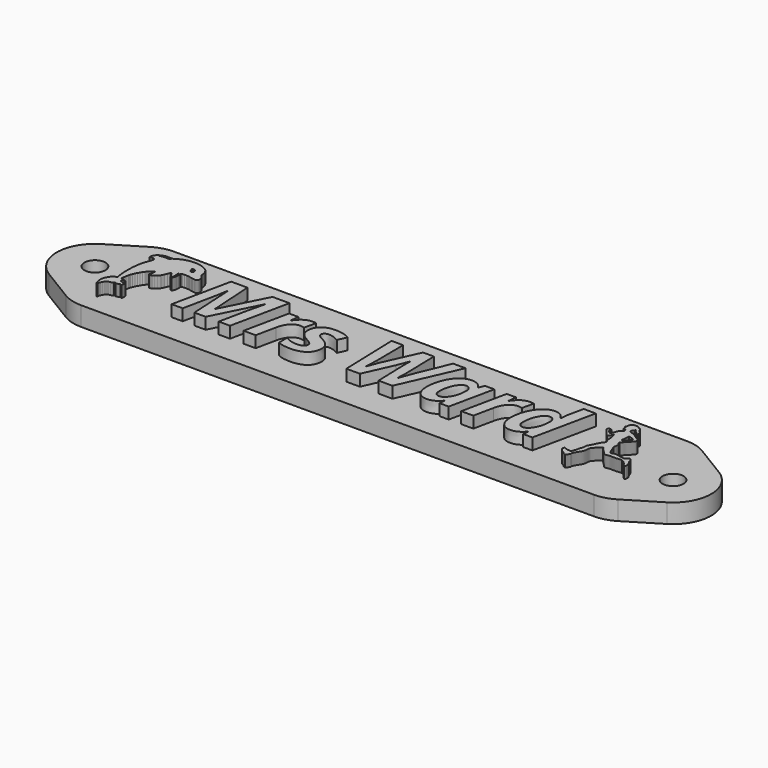
from build123d import *

# Parameters (mm, degrees)
F0_W         = 140
F0_H         = 30.4531101137
F1_DEPTH     = 5
F2_R         = 10
F3_R         = 10
F4_TEXT_SIZE = 21.5990010462
F5_DEPTH     = 3
F7_D         = 5.5
F9_DEPTH     = 3
F11_DEPTH    = 3


# Not quite as in the source:
# - Text() gives the source's letters only with a copy of the font that has no kerning and outlines rounded to 1/6400 em; it was checked with that copy


with BuildPart() as f1:
    # F0 (on Top) → F1 (new body)
    with BuildSketch(Plane.XY):
        Rectangle(F0_W, F0_H)
        Polygon((-95, 0), (-70, -15.2265550569), (-70, 15.2265550569), align=None)
        Polygon((70, 15.2265550569), (70, -15.2265550569), (95, 0), align=None)
    extrude(amount=F1_DEPTH)

    # F2
    f2_edges = [f1.edges().sort_by_distance(p)[0] for p in [
        (-95, 0, 2.5),
        (95, 0, 2.5),
    ]]
    fillet(f2_edges, radius=F2_R)

    # F3
    f3_edges = [f1.edges().sort_by_distance(p)[0] for p in [
        (70, -15.226555, 2.5),
        (-70, -15.226555, 2.5),
        (-70, 15.226555, 2.5),
        (70, 15.226555, 2.5),
    ]]
    fillet(f3_edges, radius=F3_R)

    # F4 (on face) → F5 (join)
    with BuildSketch(Plane.XY.offset(5)):
        with Locations((-50, -7.7756403766)):
            Text('Mrs Ward', F4_TEXT_SIZE, font='Open Sans', font_style=FontStyle.BOLDITALIC, text_align=(TextAlign.LEFT, TextAlign.BOTTOM))
    extrude(amount=F5_DEPTH)

    # F7 (through all)
    with Locations(Plane.XY.offset(5)):
        with Locations((75.7757134551, 0), (-75.7757134551, 0)):
            Hole(F7_D / 2)

    # F8 (on face) → F9 (join)
    with BuildSketch(Plane.XY.offset(5)):
        Polygon((-67.3505419405, -10.0196780843), (-67.2982909405, -10.0712440843), (-67.1962299405, -10.1371600843), (-67.1447409405, -10.1575460843), (-67.1015519405, -10.1654290843), (-67.0526269405, -10.1591240843), (-67.0368499405, -10.1467530843), (-67.0257719405, -10.1249220843), (-67.0144519405, -10.0429330843), (-67.0121309405, -9.8932650843), (-67.0056009405, -9.7362200843), (-66.9790779405, -9.5939760843), (-66.9221619405, -9.4281290843), (-66.8244519405, -9.2002770843), (-66.6788199405, -8.9073640843), (-66.5216759405, -8.6591190843), (-66.4371029405, -8.5505090843), (-66.3476319405, -8.4515820843), (-66.2525879405, -8.3618420843), (-66.1512979405, -8.2807950843), (-66.0430879405, -8.2079450843), (-65.9272839405, -8.1427990843), (-65.8032129405, -8.0848600843), (-65.6702019405, -8.0336340843), (-65.3746609405, -7.9493420843), (-65.0352729405, -7.8859630843), (-64.9580219405, -7.8687340843), (-64.8837989405, -7.8415260843), (-64.8148449405, -7.8060910843), (-64.7534009405, -7.7641840843), (-64.7017099405, -7.7175590843), (-64.6620119405, -7.6679700843), (-64.6365499405, -7.6171720843), (-64.6275639405, -7.5669180843), (-64.6117799405, -7.5114250843), (-64.5738299405, -7.4581930843), (-64.5419789405, -7.4398510843), (-64.5051759405, -7.4464100843), (-64.4580789405, -7.4804550843), (-64.3953489405, -7.5445710843), (-64.3244609405, -7.6145560843), (-64.2575609405, -7.6566130843), (-64.1798479405, -7.6771500843), (-64.0765239405, -7.6825720843), (-63.8993629405, -7.6648360843), (-63.7228449405, -7.6141150843), (-63.5567489405, -7.5341380843), (-63.4108539405, -7.4286390843), (-63.3037379405, -7.3480460843), (-63.2588269405, -7.3235300843), (-63.2276919405, -7.3145260843), (-63.1928879405, -7.3290540843), (-63.1379839405, -7.3686100843), (-62.9980199405, -7.4986430843), (-62.9212539405, -7.5747760843), (-62.8603179405, -7.6216400843), (-62.8125049405, -7.6359000843), (-62.7926739405, -7.6297620843), (-62.7751089405, -7.6142220843), (-62.7454209405, -7.5532720843), (-62.7207369405, -7.4497160843), (-62.6755469405, -7.1014490843), (-62.6498839405, -6.8368820843), (-62.6452669405, -6.6688380843), (-62.6644289405, -6.5419490843), (-62.7100989405, -6.4008450843), (-62.8022509405, -6.1827090843), (-62.9130539405, -5.9960690843), (-62.9768649405, -5.9135900843), (-63.0470389405, -5.8378200843), (-63.1241409405, -5.7683720843), (-63.2087379405, -5.7048560843), (-63.4026829405, -5.5940720843), (-63.6334059405, -5.5023590843), (-63.9054389405, -5.4266140843), (-64.2233139405, -5.3637290843), (-64.4953439405, -5.3079480843), (-64.5860339405, -5.2817910843), (-64.6287689405, -5.2612710843), (-64.6372809405, -5.1873330843), (-64.6270709405, -5.0232890843), (-64.5627999405, -4.5089810843), (-64.4605899405, -3.8865380843), (-64.3450719405, -3.3241520843), (-64.2861349405, -3.1009140843), (-64.2142809405, -2.8684250843), (-64.0355739405, -2.3827370843), (-63.8164509405, -1.8811740843), (-63.5644149405, -1.3778250843), (-63.2869649405, -0.8867750843), (-62.9916029405, -0.4221130843), (-62.6858299405, 0.0020739157), (-62.5313829405, 0.1945879157), (-62.3771469405, 0.3716999157), (-62.2629059405, 0.4849989157), (-62.0991469405, 0.6321189157), (-61.6979429405, 0.9674989157), (-61.3232799405, 1.2571979157), (-61.1926959405, 1.3472169157), (-61.1249019405, 1.3805739157), (-61.1111509405, 1.3725499157), (-61.1005539405, 1.3494609157), (-61.0883419405, 1.2639799157), (-61.0873009405, 1.1359229157), (-61.0964649405, 0.9770789157), (-61.1415479405, 0.6141949157), (-61.1755359405, 0.4337339157), (-61.2158679405, 0.2696489157), (-61.2729569405, 0.0548219157), (-61.3086339405, -0.1178760843), (-61.3217909405, -0.2526280843), (-61.3113189405, -0.3536200843), (-61.2761099405, -0.4250350843), (-61.2150539405, -0.4710560843), (-61.1270439405, -0.4958680843), (-61.0109709405, -0.5036550843), (-60.8371699405, -0.4895950843), (-60.6604159405, -0.4446880843), (-60.4785559405, -0.3675070843), (-60.2894359405, -0.2566240843), (-60.0909019405, -0.1106120843), (-59.8807999405, 0.0719559157), (-59.6569759405, 0.2925069157), (-59.4172759405, 0.5524699157), (-59.2193419405, 0.7841369157), (-59.0805869405, 0.9830499157), (-58.9535879405, 1.2285009157), (-58.7909259405, 1.5997829157), (-58.5557769405, 2.1779399157), (-58.3831549405, 2.6464149157), (-58.2796119405, 2.9221129157), (-58.2379389405, 3.0059819157), (-58.2105499405, 3.0367839157), (-58.1621269405, 3.0135859157), (-58.0907269405, 2.9453419157), (-57.9977919405, 2.8340759157), (-57.8847659405, 2.6818139157), (-57.6042059405, 2.2624019157), (-57.2605889405, 1.7033049157), (-57.2066639405, 1.6228809157), (-57.1472449405, 1.5518989157), (-57.0846659405, 1.4918699157), (-57.0212599405, 1.4443049157), (-56.9593609405, 1.4107149157), (-56.9013009405, 1.3926119157), (-56.8494129405, 1.3915059157), (-56.8060319405, 1.4089089157), (-56.7662869405, 1.4511629157), (-56.7176859405, 1.5248529157), (-56.6065939405, 1.7392459157), (-56.4981129405, 1.9974999157), (-56.4176029405, 2.2450299157), (-56.3909649405, 2.3735329157), (-56.3711779405, 2.5235289157), (-56.3524569405, 2.8651499157), (-56.3620359405, 3.2241999157), (-56.3776249405, 3.3959809157), (-56.4005119405, 3.5549849157), (-56.4323769405, 3.8036719157), (-56.4292449405, 3.8746809157), (-56.4135639405, 3.9145309157), (-56.3653029405, 3.9400259157), (-56.2696579405, 3.9642729157), (-55.9625549405, 4.0064239157), (-55.5449219405, 4.0357879157), (-55.0694259405, 4.0471669157), (-54.7497399405, 4.0417089157), (-54.4738059405, 4.0168859157), (-54.1592519405, 3.9615089157), (-53.7237059405, 3.8643899157), (-53.3210649405, 3.7772139157), (-52.9762069405, 3.7170829157), (-52.6850949405, 3.6841479157), (-52.4436879405, 3.6785609157), (-52.2479479405, 3.7004719157), (-52.1659409405, 3.7217859157), (-52.0938359405, 3.7500309157), (-52.0311269405, 3.7852259157), (-51.9773119405, 3.8273899157), (-51.9318829405, 3.8765409157), (-51.8943369405, 3.9326989157), (-51.8591559405, 4.0124459157), (-51.8393969405, 4.1118199157), (-51.8326569405, 4.2525939157), (-51.8365339405, 4.4565409157), (-51.8517469405, 4.6690549157), (-51.8832159405, 4.8634879157), (-51.9327739405, 5.0436279157), (-52.0022489405, 5.2132639157), (-52.0934739405, 5.3761859157), (-52.2082789405, 5.5361809157), (-52.3484949405, 5.6970399157), (-52.5159529405, 5.8625499157), (-52.7047309405, 6.0382459157), (-52.7047309405, 6.3766979157), (-52.7187109405, 6.5939379157), (-52.7587709405, 6.8284649157), (-52.8220889405, 7.0728329157), (-52.9058429405, 7.3195969157), (-53.0072099405, 7.5613079157), (-53.1233689405, 7.7905219157), (-53.2514979405, 7.9997909157), (-53.3887739405, 8.1816689157), (-53.4961709405, 8.2997909157), (-53.6135299405, 8.4134909157), (-53.7404219405, 8.5225679157), (-53.8764199405, 8.6268229157), (-54.0210959405, 8.7260559157), (-54.1740229405, 8.8200689157), (-54.5029189405, 8.9916329157), (-54.8596849405, 9.1399189157), (-55.2409009405, 9.2633309157), (-55.6431439405, 9.3602719157), (-56.0629949405, 9.4291479157), (-56.7187509405, 9.5284869157), (-56.9852389405, 9.5603269157), (-57.3064799405, 9.5678329157), (-57.6706099405, 9.5523869157), (-58.0657649405, 9.5153679157), (-58.4800789405, 9.4581589157), (-58.9016879405, 9.3821399157), (-59.3187269405, 9.2886929157), (-59.7193309405, 9.1791989157), (-59.9262099405, 9.1078689157), (-60.1692819405, 9.0093169157), (-60.7139219405, 8.7555579157), (-61.2530829405, 8.4679579157), (-61.4893069405, 8.3271019157), (-61.6865979405, 8.1965489157), (-61.7341649405, 8.1654749157), (-61.7850759405, 8.1416779157), (-61.8496709405, 8.1241809157), (-61.9382889405, 8.1120069157), (-62.2289519405, 8.0997179157), (-62.7397819405, 8.0969919157), (-63.2140199405, 8.0929199157), (-63.5504269405, 8.0790679157), (-63.8044219405, 8.0515539157), (-64.0314219405, 8.0064949157), (-64.2673049405, 7.9359229157), (-64.5124489405, 7.8363259157), (-64.7586379405, 7.7129769157), (-64.9976539405, 7.5711479157), (-65.2212809405, 7.4161139157), (-65.4212999405, 7.2531459157), (-65.5894949405, 7.0875169157), (-65.7176489405, 6.9244989157), (-65.7813429405, 6.8180659157), (-65.8442799405, 6.6950779157), (-65.9585439405, 6.4245849157), (-66.0417639405, 6.1633119157), (-66.0658959405, 6.0518479157), (-66.0752629405, 5.9615489157), (-66.0781749405, 5.7741309157), (-65.5386059405, 5.7909399157), (-65.1735809405, 5.7918459157), (-65.0419229405, 5.7803359157), (-64.9371769405, 5.7588199157), (-64.8541009405, 5.7257759157), (-64.7874529405, 5.6796799157), (-64.7319909405, 5.6190099157), (-64.6824719405, 5.5422429157), (-64.6505679405, 5.4677189157), (-64.6351609405, 5.3810069157), (-64.6374409405, 5.2766999157), (-64.6586009405, 5.1493889157), (-64.6998339405, 4.9936659157), (-64.7623309405, 4.8041229157), (-64.9558879405, 4.3019439157), (-65.1437819405, 3.8205759157), (-65.3031429405, 3.3667089157), (-65.4382029405, 2.9218309157), (-65.5531919405, 2.4674329157), (-65.6523419405, 1.9850039157), (-65.7398839405, 1.4560329157), (-65.8200489405, 0.8620099157), (-65.8970679405, 0.1844239157), (-65.9153039405, -0.0973970843), (-65.9285709405, -0.5200820843), (-65.9399899405, -1.5966640843), (-65.9309069405, -2.6625640843), (-65.9185469405, -3.0718950843), (-65.9009049405, -3.3350220843), (-65.7633849405, -4.3900910843), (-65.6972079405, -4.8097300843), (-65.6364429405, -5.1323650843), (-65.6341889405, -5.1622620843), (-65.6428699405, -5.1918550843), (-65.6658539405, -5.2238390843), (-65.7065049405, -5.2609060843), (-65.8542729405, -5.3610690843), (-66.1131009405, -5.5138950843), (-66.3849869405, -5.6762940843), (-66.5720389405, -5.8085950843), (-66.7215059405, -5.9491010843), (-66.8806389405, -6.1361180843), (-66.9936589405, -6.2874220843), (-67.1042559405, -6.4564090843), (-67.2098269405, -6.6377740843), (-67.3077699405, -6.8262100843), (-67.3954849405, -7.0164130843), (-67.4703699405, -7.2030750843), (-67.5298219405, -7.3808910843), (-67.5712409405, -7.5445560843), (-67.6171839405, -7.7360980843), (-67.6552689405, -7.8412930843), (-67.6695539405, -7.8997380843), (-67.6795589405, -8.0182590843), (-67.6869259405, -8.3600340843), (-67.6777599405, -8.7156320843), (-67.6670979405, -8.8514310843), (-67.6524489405, -8.9340660843), (-67.6150609405, -9.1033840843), (-67.5747519405, -9.3620690843), (-67.5312879405, -9.6149350843), (-67.4732199405, -9.8110170843), (-67.4375379405, -9.8907650843), (-67.3968019405, -9.9599180843), align=None)
        Polygon((-62.7648599405, -6.7480430843), (-62.7596529405, -6.8253010843), (-62.7636349405, -6.8616760843), (-62.7755099405, -6.8835840843), (-62.7951729405, -6.8910710843), (-62.8225169405, -6.8841860843), (-62.8998279405, -6.8274880843), (-63.0065979405, -6.7138720843), (-63.0638319405, -6.6548840843), (-63.1322849405, -6.5986590843), (-63.3013009405, -6.4952870843), (-63.5105489405, -6.4053380843), (-63.7569339405, -6.3303930843), (-63.8070529405, -6.3104920843), (-63.8598369405, -6.2771980843), (-63.9618759405, -6.1833790843), (-64.0400009405, -6.0748230843), (-64.0628939405, -6.0231100843), (-64.0711649405, -5.9774220843), (-64.0625409405, -5.9375650843), (-64.0390599405, -5.8899530843), (-64.0043089405, -5.8405610843), (-63.9618729405, -5.7953630843), (-63.8986189405, -5.7455820843), (-63.8367459405, -5.7196300843), (-63.7613649405, -5.7140930843), (-63.6575869405, -5.7255530843), (-63.4837859405, -5.7651630843), (-63.4104709405, -5.7951330843), (-63.3419399405, -5.8347500843), (-63.2749889405, -5.8861680843), (-63.2064149405, -5.9515390843), (-63.0515769405, -6.1327540843), (-62.9304949405, -6.3087350843), (-62.8385319405, -6.4898150843), (-62.7801099405, -6.6655010843), align=None, mode=Mode.SUBTRACT)
        Polygon((-67.1281399405, -9.2141380843), (-67.1613879405, -9.4302710843), (-67.1787649405, -9.5439900843), (-67.1997019405, -9.6251770843), (-67.2247949405, -9.6755320843), (-67.2546379405, -9.6967570843), (-67.2779179405, -9.6849700843), (-67.3020009405, -9.6388550843), (-67.3532069405, -9.4404540843), (-67.4095169405, -9.0951840843), (-67.4721889405, -8.5966740843), (-67.4806749405, -8.4699190843), (-67.4786139405, -8.3333960843), (-67.4449569405, -8.0370070843), (-67.3754279405, -7.7194330843), (-67.2742359405, -7.3925950843), (-67.1455909405, -7.0684170843), (-66.9937009405, -6.7588240843), (-66.8227779405, -6.4757390843), (-66.7314929405, -6.3478630843), (-66.6370289405, -6.2310850843), (-66.5469939405, -6.1378330843), (-66.4448909405, -6.0518230843), (-66.3313829405, -5.9733970843), (-66.2071339405, -5.9028930843), (-66.0728069405, -5.8406540843), (-65.9290659405, -5.7870190843), (-65.7765719405, -5.7423290843), (-65.6159899405, -5.7069240843), (-65.4380379405, -5.6681740843), (-65.3526079405, -5.6388430843), (-65.3567219405, -5.5243140843), (-65.3940569405, -5.2807240843), (-65.5273219405, -4.5322530843), (-65.6129099405, -4.0008260843), (-65.6668119405, -3.5769180843), (-65.7050199405, -3.1510000843), (-65.7355159405, -2.6462120843), (-65.7525539405, -2.1122670843), (-65.7565499405, -1.5643830843), (-65.7479209405, -1.0177770843), (-65.7270819405, -0.4876670843), (-65.6944509405, 0.0107289157), (-65.6504439405, 0.4621929157), (-65.5954779405, 0.8515069157), (-65.5349659405, 1.1682439157), (-65.4505829405, 1.5584709157), (-65.2389119405, 2.4450219157), (-65.0178819405, 3.2824099157), (-64.9217979405, 3.6111839157), (-64.8449049405, 3.8418859157), (-64.7435149405, 4.1179209157), (-64.4840369405, 4.7850059157), (-64.3230309405, 5.2278459157), (-64.2735179405, 5.4015369157), (-64.2438819405, 5.5487269157), (-64.2335379405, 5.6734029157), (-64.2418979405, 5.7795529157), (-64.2683769405, 5.8711649157), (-64.3123879405, 5.9522269157), (-64.3652219405, 6.0204769157), (-64.4237099405, 6.0766249157), (-64.4904489405, 6.1215959157), (-64.5680319405, 6.1563159157), (-64.6590559405, 6.1817089157), (-64.7661149405, 6.1987019157), (-65.0387209405, 6.2111859157), (-65.2171249405, 6.2160979157), (-65.3506039405, 6.2328449157), (-65.4405349405, 6.2644419157), (-65.4695999405, 6.2867499157), (-65.4882949405, 6.3139019157), (-65.4967919405, 6.3462729157), (-65.4952619405, 6.3842399157), (-65.4628109405, 6.4784719157), (-65.3923219405, 6.5996119157), (-65.2851699405, 6.7506739157), (-65.1976099405, 6.8533129157), (-65.0962069405, 6.9468159157), (-64.9828869405, 7.0301819157), (-64.8595759405, 7.1024109157), (-64.7281959405, 7.1625029157), (-64.5906749405, 7.2094579157), (-64.4489359405, 7.2422759157), (-64.3049039405, 7.2599569157), (-64.1720429405, 7.2641819157), (-64.0466589405, 7.2593409157), (-63.9387799405, 7.2462069157), (-63.8584369405, 7.2255519157), (-63.7948539405, 7.1914499157), (-63.7256079405, 7.1380009157), (-63.5875599405, 6.9943429157), (-63.4791619405, 6.8371429157), (-63.4469769405, 6.7667679157), (-63.4352809405, 6.7089689157), (-63.4249249405, 6.6426109157), (-63.4102359405, 6.6324549157), (-63.3876559405, 6.6384709157), (-63.3141689405, 6.7014969157), (-63.1951629405, 6.8366329157), (-63.0738069405, 6.9716189157), (-62.9466889405, 7.0961229157), (-62.8205709405, 7.2054449157), (-62.7022169405, 7.2948899157), (-62.5983909405, 7.3597589157), (-62.5158559405, 7.3953549157), (-62.4846859405, 7.4007079157), (-62.4613749405, 7.3969809157), (-62.4467679405, 7.3835869157), (-62.4417109405, 7.3599389157), (-62.4743819405, 7.2976849157), (-62.5633359405, 7.1632229157), (-62.8557529405, 6.7568279157), (-63.1686279405, 6.3244989157), (-63.4365529405, 5.9268779157), (-63.6654519405, 5.5547899157), (-63.8612459405, 5.1990579157), (-64.0380669405, 4.7994149157), (-64.2632769405, 4.2219299157), (-64.4740909405, 3.6343669157), (-64.6077239405, 3.2044869157), (-64.6568779405, 2.9723689157), (-64.6608489405, 2.9159619157), (-64.6522329405, 2.8990969157), (-64.6318909405, 2.9216079157), (-64.6006849405, 2.9833269157), (-64.5091279405, 3.2237129157), (-64.3130649405, 3.7417009157), (-64.0570219405, 4.3507679157), (-63.7936589405, 4.9303989157), (-63.5756359405, 5.3600779157), (-63.4543819405, 5.5619009157), (-63.3070439405, 5.7866789157), (-62.9635069405, 6.2660809157), (-62.6038079405, 6.7202459157), (-62.4362659405, 6.9134789157), (-62.2867279405, 7.0711389157), (-62.0690659405, 7.2771519157), (-61.8419359405, 7.4739969157), (-61.6057509405, 7.6614769157), (-61.3609239405, 7.8393939157), (-61.1078709405, 8.0075529157), (-60.8470049405, 8.1657559157), (-60.5787389405, 8.3138069157), (-60.3034879405, 8.4515079157), (-60.0216659405, 8.5786639157), (-59.7336869405, 8.6950759157), (-59.4399639405, 8.8005489157), (-59.1409109405, 8.8948859157), (-58.8369429405, 8.9778889157), (-58.5284729405, 9.0493629157), (-58.2159159405, 9.1091089157), (-57.8996839405, 9.1569319157), (-57.5912779405, 9.1873959157), (-57.2538059405, 9.2029479157), (-56.8988669405, 9.2042019157), (-56.5380609405, 9.1917729157), (-56.1829859405, 9.1662759157), (-55.8452419405, 9.1283239157), (-55.5364269405, 9.0785319157), (-55.2681399405, 9.0175149157), (-54.9778939405, 8.9257489157), (-54.6850409405, 8.8095629157), (-54.3984699405, 8.6742199157), (-54.1270679405, 8.5249809157), (-53.8797239405, 8.3671079157), (-53.6653259405, 8.2058639157), (-53.4927619405, 8.0465109157), (-53.4249459405, 7.9691879157), (-53.3709209405, 7.8943109157), (-53.2994699405, 7.7713639157), (-53.2250659405, 7.6246919157), (-53.0824759405, 7.2981599157), (-52.9733159405, 6.9906769157), (-52.9406979405, 6.8678179157), (-52.9277479405, 6.7782069157), (-52.9294679405, 6.6941319157), (-52.9392239405, 6.6361859157), (-52.9561429405, 6.6041519157), (-52.9793509405, 6.5978139157), (-53.0079759405, 6.6169559157), (-53.0411419405, 6.6613639157), (-53.1176109405, 6.8251109157), (-53.1862329405, 6.9809449157), (-53.2775559405, 7.1552979157), (-53.4928429405, 7.5067079157), (-53.5990719405, 7.6573419157), (-53.6925359405, 7.7736459157), (-53.7643689405, 7.8424079157), (-53.7894019405, 7.8548309157), (-53.8057029405, 7.8504149157), (-53.7953159405, 7.8076699157), (-53.7523529405, 7.7082829157), (-53.5961959405, 7.3988519157), (-53.4710309405, 7.1540439157), (-53.3717649405, 6.9351119157), (-53.2980309405, 6.7404179157), (-53.2494629405, 6.5683229157), (-53.2256939405, 6.4171889157), (-53.2263579405, 6.2853779157), (-53.2510879405, 6.1712499157), (-53.2995169405, 6.0731689157), (-53.3504849405, 6.0093579157), (-53.3801059405, 5.9892679157), (-53.4183559405, 5.9756169157), (-53.5383639405, 5.9633099157), (-53.7457399405, 5.9638009157), (-53.9163519405, 5.9712969157), (-54.0665429405, 5.9880069157), (-54.1935079405, 6.0135039157), (-54.2944409405, 6.0473599157), (-54.5577109405, 6.1527629157), (-54.6018179405, 6.1556239157), (-54.6123839405, 6.1318519157), (-54.5959209405, 6.1041839157), (-54.5510929405, 6.0614229157), (-54.4037339405, 5.9539639157), (-54.2727749405, 5.8770839157), (-54.2105749405, 5.8533179157), (-54.1373599405, 5.8372989157), (-53.9182799405, 5.8223899157), (-53.5363259405, 5.8201369157), (-52.8775669405, 5.8201369157), (-52.7271379405, 5.6873969157), (-52.4835599405, 5.4647289157), (-52.2906619405, 5.2703869157), (-52.1470339405, 5.1017389157), (-52.0512629405, 4.9561489157), (-52.0208829405, 4.8911779157), (-52.0019379405, 4.8309839157), (-51.9942519405, 4.7752389157), (-51.9976469405, 4.7236109157), (-52.0119489405, 4.6757729157), (-52.0369799405, 4.6313959157), (-52.0725639405, 4.5901489157), (-52.1185239405, 4.5517039157), (-52.1952229405, 4.5041289157), (-52.2737609405, 4.4797799157), (-52.3757149405, 4.4751969157), (-52.5226599405, 4.4869219157), (-52.7761789405, 4.5332199157), (-52.8994659405, 4.5673129157), (-52.9995729405, 4.6035969157), (-53.1019369405, 4.6564979157), (-53.2353759405, 4.7377989157), (-53.5509719405, 4.9534999157), (-53.8573519405, 5.1864889157), (-53.9792699405, 5.2894009157), (-54.0655059405, 5.3725549157), (-54.1486359405, 5.4492629157), (-54.1787769405, 5.4669819157), (-54.1956089405, 5.4668179157), (-54.1795499405, 5.4317899157), (-54.1162999405, 5.3589849157), (-53.8909879405, 5.1395049157), (-53.6052029405, 4.8873119157), (-53.3444729405, 4.6813359157), (-53.2048659405, 4.5731679157), (-53.1221729405, 4.4897179157), (-53.1033609405, 4.4588229157), (-53.1002079405, 4.4359819157), (-53.1131889405, 4.4218189157), (-53.1427829405, 4.4169589157), (-53.1982549405, 4.4339569157), (-53.2933139405, 4.4812119157), (-53.5667679405, 4.6440479157), (-53.8922809405, 4.8605849157), (-54.1989919405, 5.0859399157), (-54.5145139405, 5.3249669157), (-54.7338539405, 5.4764159157), (-54.8119889405, 5.5144339157), (-54.9060329405, 5.5480639157), (-55.1066579405, 5.5962029157), (-55.1956419405, 5.6077319157), (-55.2653449405, 5.6089149157), (-55.3069679405, 5.5982599157), (-55.3144999405, 5.5880289157), (-55.3117129405, 5.5742789157), (-55.2913609405, 5.5536299157), (-55.2569379405, 5.5367199157), (-55.1651159405, 5.5210989157), (-55.1049629405, 5.5135889157), (-55.0331629405, 5.4918569157), (-54.8630269405, 5.4104939157), (-54.6715209405, 5.2865539157), (-54.4754549405, 5.1295819157), (-54.2279279405, 4.9237369157), (-53.9560489405, 4.7194749157), (-53.6835509405, 4.5337939157), (-53.4341649405, 4.3836939157), (-53.3264259405, 4.3301949157), (-53.2047719405, 4.2803559157), (-52.9272039405, 4.1936089157), (-52.6164319405, 4.1273479157), (-52.2874309405, 4.0854649157), (-52.1751579405, 4.0639859157), (-52.1410039405, 4.0481819157), (-52.1284599405, 4.0313699157), (-52.1410269405, 3.9959619157), (-52.1759759405, 3.9595609157), (-52.2291819405, 3.9239309157), (-52.2965179405, 3.8908379157), (-52.4570719405, 3.8393239157), (-52.5420369405, 3.8244329157), (-52.6246249405, 3.8191399157), (-52.7311939405, 3.8223279157), (-52.8309649405, 3.8332419157), (-52.9305629405, 3.8543039157), (-53.0366149405, 3.8879329157), (-53.2945899405, 4.0025749157), (-53.6579029405, 4.1965299157), (-54.0381399405, 4.4013299157), (-54.3710979405, 4.5664959157), (-54.6693989405, 4.6959129157), (-54.9456659405, 4.7934639157), (-55.2125229405, 4.8630339157), (-55.4825929405, 4.9085069157), (-55.7684999405, 4.9337679157), (-56.0828659405, 4.9426999157), (-56.3863199405, 4.9400059157), (-56.6157329405, 4.9206959157), (-56.8412889405, 4.8746949157), (-57.1331699405, 4.7919289157), (-57.6995039405, 4.6144849157), (-57.7354229405, 4.6068339157), (-57.7541379405, 4.6212719157), (-57.7569879405, 4.6539589157), (-57.7453119405, 4.7010549157), (-57.6837399405, 4.8231159157), (-57.5801359405, 4.9567389157), (-57.5026949405, 5.0262679157), (-57.3971659405, 5.1028849157), (-57.1394159405, 5.2572169157), (-56.8820319405, 5.3793969157), (-56.7769609405, 5.4158239157), (-56.7001619405, 5.4290869157), (-56.6681379405, 5.4329129157), (-56.6485079405, 5.4437229157), (-56.6408679405, 5.4605129157), (-56.6448159405, 5.4822809157), (-56.6858639405, 5.5367389157), (-56.7684289405, 5.5990729157), (-56.8614629405, 5.6344599157), (-57.0067209405, 5.6633629157), (-57.1886109405, 5.6850619157), (-57.3915439405, 5.6988409157), (-57.5999289405, 5.7039819157), (-57.7981769405, 5.6997689157), (-57.9706959405, 5.6854849157), (-58.1018979405, 5.6604119157), (-58.2894509405, 5.5945429157), (-58.4723689405, 5.5129909157), (-58.6111129405, 5.4353249157), (-58.6515649405, 5.4040659157), (-58.6661469405, 5.3811159157), (-58.6407769405, 5.3669969157), (-58.5717009405, 5.3556389157), (-58.3446289405, 5.3458379157), (-58.1052639405, 5.3325689157), (-58.0228809405, 5.3174569157), (-57.9812619405, 5.2987549157), (-57.9749499405, 5.2635549157), (-58.0010779405, 5.2070829157), (-58.0613069405, 5.1267069157), (-58.1572979405, 5.0197929157), (-58.2815009405, 4.8773069157), (-58.3891179405, 4.7243739157), (-58.4854529405, 4.5466419157), (-58.5758079405, 4.3297619157), (-58.6654839405, 4.0593829157), (-58.7597849405, 3.7211549157), (-58.9834639405, 2.7837519157), (-59.1047599405, 2.2618249157), (-59.2127939405, 1.8476719157), (-59.3193669405, 1.5184869157), (-59.3757929405, 1.3786319157), (-59.4362789405, 1.2514669157), (-59.5022989405, 1.1341419157), (-59.5753279405, 1.0238059157), (-59.7483149405, 0.8126989157), (-59.9670399405, 0.5953419157), (-60.2433019405, 0.3489299157), (-60.5531189405, 0.0882489157), (-60.7579599405, -0.0574880843), (-60.8315299405, -0.0933440843), (-60.8914739405, -0.1077750843), (-60.9419989405, -0.1032180843), (-60.9873109405, -0.0821080843), (-61.0169019405, -0.0585410843), (-61.0361109405, -0.0299500843), (-61.0442799405, 0.0076759157), (-61.0407519405, 0.0583449157), (-60.9959769405, 0.2148509157), (-60.8965259405, 0.4716429157), (-60.7882789405, 0.7514279157), (-60.7027519405, 1.0040499157), (-60.6382929405, 1.2401439157), (-60.5932459405, 1.4703429157), (-60.5659579405, 1.7052829157), (-60.5547759405, 1.9555969157), (-60.5580449405, 2.2319209157), (-60.5741119405, 2.5448879157), (-60.6150899405, 2.9758989157), (-60.6765689405, 3.3226369157), (-60.7153089405, 3.4657289157), (-60.7595479405, 3.5893409157), (-60.8094119405, 3.6940059157), (-60.8650239405, 3.7802509157), (-60.9407409405, 3.8947309157), (-60.9588729405, 3.9420549157), (-60.9636689405, 3.9871149157), (-60.9549889405, 4.0331679157), (-60.9326959405, 4.0834729157), (-60.8467109405, 4.2098769157), (-60.7638399405, 4.3316879157), (-60.7425759405, 4.3733109157), (-60.7394519405, 4.3940219157), (-60.7744959405, 4.3855509157), (-60.8527119405, 4.3418449157), (-61.0972789405, 4.1780269157), (-61.3903959405, 3.9611599157), (-61.6493079405, 3.7498379157), (-61.9339079405, 3.4802129157), (-62.2038889405, 3.1904949157), (-62.4359319405, 2.9072979157), (-62.6067149405, 2.6572359157), (-62.7284249405, 2.4704089157), (-62.7744819405, 2.4135759157), (-62.8021249405, 2.3927029157), (-62.8335449405, 2.4008259157), (-62.8527429405, 2.4256549157), (-62.8596019405, 2.4678769157), (-62.8540039405, 2.5281789157), (-62.8049709405, 2.7057769157), (-62.7047029405, 2.9639489157), (-62.5967189405, 3.2067409157), (-62.4950789405, 3.3859999157), (-62.3655749405, 3.5529679157), (-62.1739959405, 3.7588879157), (-61.8382909405, 4.0958589157), (-61.5483469405, 4.3551129157), (-61.2432119405, 4.5869499157), (-60.8619359405, 4.8416709157), (-60.7145769405, 4.9424979157), (-60.6532859405, 4.9963639157), (-60.6589129405, 5.0052139157), (-60.6754749405, 5.0075979157), (-60.7394869405, 4.9938359157), (-60.9776539405, 4.8982579157), (-61.3371359405, 4.7234949157), (-61.7872819405, 4.4834099157), (-61.9137819405, 4.4031059157), (-62.0636799405, 4.2910469157), (-62.4010699405, 4.0016069157), (-62.7342619405, 3.6749829157), (-62.8789109405, 3.5164429157), (-62.9980639405, 3.3710649157), (-63.3066049405, 2.9329769157), (-63.6320359405, 2.4175539157), (-63.9313949405, 1.8960949157), (-64.0578719405, 1.6553829157), (-64.1617209405, 1.4398989157), (-64.3221559405, 1.0220269157), (-64.5400819405, 0.3838379157), (-64.7518999405, -0.2817200843), (-64.8940089405, -0.7816990843), (-65.0923899405, -1.7018160843), (-65.1660709405, -2.0820240843), (-65.2079849405, -2.3799910843), (-65.2276519405, -2.6896650843), (-65.2345939405, -3.1049920843), (-65.2308019405, -3.6680810843), (-65.2114259405, -4.0977900843), (-65.1784589405, -4.3674810843), (-65.1575019405, -4.4339940843), (-65.1460149405, -4.4487110843), (-65.1338949405, -4.4505130843), (-65.1117699405, -4.4259040843), (-65.0835189405, -4.3712410843), (-65.0231679405, -4.2041000843), (-64.9461419405, -3.9659980843), (-64.8764469405, -3.8024440843), (-64.8439879405, -3.7479320843), (-64.8129279405, -3.7112280843), (-64.7831229405, -3.6920570843), (-64.7544289405, -3.6901420843), (-64.7296909405, -3.6959510843), (-64.7119419405, -3.7076990843), (-64.7010639405, -3.7367960843), (-64.6969389405, -3.7946490843), (-64.7084739405, -4.0422580843), (-64.7455999405, -4.5417910843), (-64.7700139405, -4.9709230843), (-64.7655719405, -5.2965230843), (-64.7514259405, -5.4365310843), (-64.7287399405, -5.5698940843), (-64.6559829405, -5.8423400843), (-64.5891469405, -6.0363480843), (-64.5223249405, -6.1909600843), (-64.4463519405, -6.3246830843), (-64.3520609405, -6.4560240843), (-64.2950949405, -6.5230660843), (-64.2354479405, -6.5804470843), (-64.1705289405, -6.6294660843), (-64.0977439405, -6.6714210843), (-64.0145019405, -6.7076110843), (-63.9182099405, -6.7393330843), (-63.6761059405, -6.7945720843), (-63.4358059405, -6.8549710843), (-63.2315819405, -6.9369510843), (-63.1470529405, -6.9840130843), (-63.0764079405, -7.0340470843), (-63.0212689405, -7.0862450843), (-62.9832559405, -7.1397980843), (-62.9566929405, -7.2097800843), (-62.9595639405, -7.2305650843), (-62.9734639405, -7.2419690843), (-63.0351269405, -7.2369050843), (-63.1432409405, -7.1951250843), (-63.2375069405, -7.1570250843), (-63.3132109405, -7.1488520843), (-63.4025659405, -7.1739020843), (-63.5377839405, -7.2354680843), (-63.7358779405, -7.3238620843), (-63.8817089405, -7.3780570843), (-63.9399449405, -7.3831040843), (-64.0167889405, -7.3737410843), (-64.2040589405, -7.3199720843), (-64.3990339405, -7.2331150843), (-64.4855089405, -7.1823940843), (-64.5572269405, -7.1295370843), (-64.6657319405, -7.0370850843), (-64.7220499405, -7.1931120843), (-64.7608009405, -7.2696100843), (-64.8202719405, -7.3419580843), (-64.9003519405, -7.4100930843), (-65.0009289405, -7.4739530843), (-65.1218909405, -7.5334750843), (-65.2631249405, -7.5885980843), (-65.4245199405, -7.6392580843), (-65.6059629405, -7.6853940843), (-65.9240759405, -7.7704210843), (-66.1374109405, -7.8485120843), (-66.2325129405, -7.9067310843), (-66.3343819405, -7.9834500843), (-66.5441639405, -8.1776300843), (-66.7382549405, -8.4015460843), (-66.8205079405, -8.5154340843), (-66.8881499405, -8.6256900843), (-67.0036199405, -8.8474770843), (-67.0795839405, -9.0317500843), align=None, mode=Mode.SUBTRACT)
        Polygon((-64.0437169405, -1.6077120843), (-64.2382239405, -1.9734530843), (-64.2931919405, -2.0668800843), (-64.3415699405, -2.1103500843), (-64.3609869405, -2.1124080843), (-64.3759959405, -2.1008440843), (-64.3856759405, -2.0752810843), (-64.3891069405, -2.0353410843), (-64.3740329405, -1.9052310843), (-64.3359999405, -1.6829570843), (-64.2342019405, -1.1957520843), (-64.1576079405, -0.8737100843), (-64.0989389405, -0.6480580843), (-64.0238069405, -0.4037630843), (-63.8346319405, 0.1145309157), (-63.6110509405, 0.6287239157), (-63.4929099405, 0.8678929157), (-63.3740299405, 1.0863679157), (-63.2578769405, 1.2732369157), (-63.1127169405, 1.4832919157), (-62.7724359405, 1.9273329157), (-62.4273069405, 2.3272279157), (-62.2760859405, 2.4821009157), (-62.1514479405, 2.5917159157), (-61.8933749405, 2.7709289157), (-61.5843219405, 2.9615749157), (-61.3104819405, 3.1130629157), (-61.2137019405, 3.1583129157), (-61.1580469405, 3.1748019157), (-61.1269539405, 3.1649809157), (-61.0909059405, 3.1382399157), (-61.0543719405, 3.0986649157), (-61.0218229405, 3.0503379157), (-60.9908499405, 2.9593879157), (-60.9678809405, 2.8208509157), (-60.9531049405, 2.6511999157), (-60.9467119405, 2.4669089157), (-60.9488919405, 2.2844519157), (-60.9598319405, 2.1203009157), (-60.9797239405, 1.9909289157), (-61.0087549405, 1.9128109157), (-61.0551399405, 1.8676699157), (-61.1390049405, 1.8039989157), (-61.3715579405, 1.6549199157), (-61.5714789405, 1.5257019157), (-61.7783539405, 1.3664129157), (-61.9931679405, 1.1760259157), (-62.2169019405, 0.9535119157), (-62.4505409405, 0.6978429157), (-62.6950679405, 0.4079919157), (-62.9514649405, 0.0829299157), (-63.2207169405, -0.2783700843), (-63.4637469405, -0.6415290843), (-63.7618199405, -1.1241900843), align=None, mode=Mode.SUBTRACT)
        Polygon((-56.6531959405, 2.0592149157), (-56.7034579405, 1.9807419157), (-56.7918589405, 1.8817899157), (-56.8315719405, 1.8516879157), (-56.8613829405, 1.8406329157), (-56.8855239405, 1.8475349157), (-56.9026159405, 1.8663419157), (-56.9157819405, 1.9282759157), (-56.9011289405, 2.0036429157), (-56.8834469405, 2.0392409157), (-56.8589019405, 2.0696519157), (-56.8235649405, 2.1153779157), (-56.7975929405, 2.1766719157), (-56.7809469405, 2.2550909157), (-56.7735859405, 2.3521899157), (-56.7865639405, 2.6086549157), (-56.8362079405, 2.9585139157), (-56.8894459405, 3.3365629157), (-56.8969569405, 3.4703699157), (-56.8910419405, 3.5720199157), (-56.8711849405, 3.6450039157), (-56.8368719405, 3.6928129157), (-56.7875879405, 3.7189389157), (-56.7228159405, 3.7268719157), (-56.6693439405, 3.7188949157), (-56.6255479405, 3.6927459157), (-56.5905159405, 3.6450949157), (-56.5633369405, 3.5726119157), (-56.5430979405, 3.4719679157), (-56.5288869405, 3.3398339157), (-56.5149049405, 2.9677759157), (-56.5208219405, 2.6202759157), (-56.5517999405, 2.3526079157), (-56.5778209405, 2.2427719157), (-56.6114679405, 2.1457659157), align=None, mode=Mode.SUBTRACT)
        Polygon((-64.0701939405, 7.5093469157), (-64.2698789405, 7.4754199157), (-64.6017779405, 7.4049779157), (-64.7945249405, 7.3717139157), (-64.8839209405, 7.3713639157), (-64.9010489405, 7.3821979157), (-64.9057639405, 7.3996609157), (-64.8971709405, 7.4247009157), (-64.8723149405, 7.4529059157), (-64.7793419405, 7.5167449157), (-64.6378999405, 7.5870479157), (-64.4590489405, 7.6596839157), (-64.2538449405, 7.7305219157), (-64.0333469405, 7.7954319157), (-63.8086109405, 7.8502819157), (-63.5906959405, 7.8909409157), (-63.3842769405, 7.9162889157), (-63.1446089405, 7.9360139157), (-62.6382909405, 7.9573209157), (-62.2172729405, 7.9523049157), (-62.0842299405, 7.9391279157), (-62.0450339405, 7.9297309157), (-62.0270859405, 7.9184109157), (-62.0311979405, 7.8893039157), (-62.0585739405, 7.8403609157), (-62.1650129405, 7.7102779157), (-62.3248269405, 7.5431429157), (-63.1284459405, 7.5462379157), (-63.5175939405, 7.5436319157), (-63.8254709405, 7.5317099157), align=None, mode=Mode.SUBTRACT)
        Polygon((-67.1787649405, -9.5439900843), (-67.1613879405, -9.4302710843), (-67.1281399405, -9.2141380843), (-67.0795839405, -9.0317500843), (-67.0036199405, -8.8474770843), (-66.8881499405, -8.6256900843), (-66.8205079405, -8.5154340843), (-66.7382549405, -8.4015460843), (-66.5441639405, -8.1776300843), (-66.3343819405, -7.9834500843), (-66.2325129405, -7.9067310843), (-66.1374109405, -7.8485120843), (-65.9240759405, -7.7704210843), (-65.6059629405, -7.6853940843), (-65.4245199405, -7.6392580843), (-65.2631249405, -7.5885980843), (-65.1218909405, -7.5334750843), (-65.0009289405, -7.4739530843), (-64.9003519405, -7.4100930843), (-64.8202719405, -7.3419580843), (-64.7608009405, -7.2696100843), (-64.7220499405, -7.1931120843), (-64.6657319405, -7.0370850843), (-64.5572269405, -7.1295370843), (-64.4855089405, -7.1823940843), (-64.3990339405, -7.2331150843), (-64.2040589405, -7.3199720843), (-64.0167889405, -7.3737410843), (-63.9399449405, -7.3831040843), (-63.8817089405, -7.3780570843), (-63.7358779405, -7.3238620843), (-63.5377839405, -7.2354680843), (-63.4025659405, -7.1739020843), (-63.3132109405, -7.1488520843), (-63.2375069405, -7.1570250843), (-63.1432409405, -7.1951250843), (-63.0351269405, -7.2369050843), (-62.9734639405, -7.2419690843), (-62.9595639405, -7.2305650843), (-62.9566929405, -7.2097800843), (-62.9832559405, -7.1397980843), (-63.0212689405, -7.0862450843), (-63.0764079405, -7.0340470843), (-63.1470529405, -6.9840130843), (-63.2315819405, -6.9369510843), (-63.4358059405, -6.8549710843), (-63.6761059405, -6.7945720843), (-63.9182099405, -6.7393330843), (-64.0145019405, -6.7076110843), (-64.0977439405, -6.6714210843), (-64.1705289405, -6.6294660843), (-64.2354479405, -6.5804470843), (-64.2950949405, -6.5230660843), (-64.3520609405, -6.4560240843), (-64.4463519405, -6.3246830843), (-64.5223249405, -6.1909600843), (-64.5891469405, -6.0363480843), (-64.6559829405, -5.8423400843), (-64.7287399405, -5.5698940843), (-64.7514259405, -5.4365310843), (-64.7655719405, -5.2965230843), (-64.7700139405, -4.9709230843), (-64.7455999405, -4.5417910843), (-64.7084739405, -4.0422580843), (-64.6969389405, -3.7946490843), (-64.7010639405, -3.7367960843), (-64.7119419405, -3.7076990843), (-64.7296909405, -3.6959510843), (-64.7544289405, -3.6901420843), (-64.7831229405, -3.6920570843), (-64.8129279405, -3.7112280843), (-64.8439879405, -3.7479320843), (-64.8764469405, -3.8024440843), (-64.9461419405, -3.9659980843), (-65.0231679405, -4.2041000843), (-65.0835189405, -4.3712410843), (-65.1117699405, -4.4259040843), (-65.1338949405, -4.4505130843), (-65.1460149405, -4.4487110843), (-65.1575019405, -4.4339940843), (-65.1784589405, -4.3674810843), (-65.2114259405, -4.0977900843), (-65.2308019405, -3.6680810843), (-65.2345939405, -3.1049920843), (-65.2276519405, -2.6896650843), (-65.2079849405, -2.3799910843), (-65.1660709405, -2.0820240843), (-65.0923899405, -1.7018160843), (-64.8940089405, -0.7816990843), (-64.7518999405, -0.2817200843), (-64.5400819405, 0.3838379157), (-64.3221559405, 1.0220269157), (-64.1617209405, 1.4398989157), (-64.0578719405, 1.6553829157), (-63.9313949405, 1.8960949157), (-63.6320359405, 2.4175539157), (-63.3066049405, 2.9329769157), (-62.9980639405, 3.3710649157), (-62.8789109405, 3.5164429157), (-62.7342619405, 3.6749829157), (-62.4010699405, 4.0016069157), (-62.0636799405, 4.2910469157), (-61.9137819405, 4.4031059157), (-61.7872819405, 4.4834099157), (-61.3371359405, 4.7234949157), (-60.9776539405, 4.8982579157), (-60.7394869405, 4.9938359157), (-60.6754749405, 5.0075979157), (-60.6589129405, 5.0052139157), (-60.6532859405, 4.9963639157), (-60.7145769405, 4.9424979157), (-60.8619359405, 4.8416709157), (-61.2432119405, 4.5869499157), (-61.5483469405, 4.3551129157), (-61.8382909405, 4.0958589157), (-62.1739959405, 3.7588879157), (-62.3655749405, 3.5529679157), (-62.4950789405, 3.3859999157), (-62.5967189405, 3.2067409157), (-62.7047029405, 2.9639489157), (-62.8049709405, 2.7057769157), (-62.8540039405, 2.5281789157), (-62.8596019405, 2.4678769157), (-62.8527429405, 2.4256549157), (-62.8335449405, 2.4008259157), (-62.8021249405, 2.3927029157), (-62.7744819405, 2.4135759157), (-62.7284249405, 2.4704089157), (-62.6067149405, 2.6572359157), (-62.4359319405, 2.9072979157), (-62.2038889405, 3.1904949157), (-61.9339079405, 3.4802129157), (-61.6493079405, 3.7498379157), (-61.3903959405, 3.9611599157), (-61.0972789405, 4.1780269157), (-60.8527119405, 4.3418449157), (-60.7744959405, 4.3855509157), (-60.7394519405, 4.3940219157), (-60.7425759405, 4.3733109157), (-60.7638399405, 4.3316879157), (-60.8467109405, 4.2098769157), (-60.9326959405, 4.0834729157), (-60.9549889405, 4.0331679157), (-60.9636689405, 3.9871149157), (-60.9588729405, 3.9420549157), (-60.9407409405, 3.8947309157), (-60.8650239405, 3.7802509157), (-60.8094119405, 3.6940059157), (-60.7595479405, 3.5893409157), (-60.7153089405, 3.4657289157), (-60.6765689405, 3.3226369157), (-60.6150899405, 2.9758989157), (-60.5741119405, 2.5448879157), (-60.5580449405, 2.2319209157), (-60.5547759405, 1.9555969157), (-60.5659579405, 1.7052829157), (-60.5932459405, 1.4703429157), (-60.6382929405, 1.2401439157), (-60.7027519405, 1.0040499157), (-60.7882789405, 0.7514279157), (-60.8965259405, 0.4716429157), (-60.9959769405, 0.2148509157), (-61.0407519405, 0.0583449157), (-61.0442799405, 0.0076759157), (-61.0361109405, -0.0299500843), (-61.0169019405, -0.0585410843), (-60.9873109405, -0.0821080843), (-60.9419989405, -0.1032180843), (-60.8914739405, -0.1077750843), (-60.8315299405, -0.0933440843), (-60.7579599405, -0.0574880843), (-60.5531189405, 0.0882489157), (-60.2433019405, 0.3489299157), (-59.9670399405, 0.5953419157), (-59.7483149405, 0.8126989157), (-59.5753279405, 1.0238059157), (-59.5022989405, 1.1341419157), (-59.4362789405, 1.2514669157), (-59.3757929405, 1.3786319157), (-59.3193669405, 1.5184869157), (-59.2127939405, 1.8476719157), (-59.1047599405, 2.2618249157), (-58.9834639405, 2.7837519157), (-58.7597849405, 3.7211549157), (-58.6654839405, 4.0593829157), (-58.5758079405, 4.3297619157), (-58.4854529405, 4.5466419157), (-58.3891179405, 4.7243739157), (-58.2815009405, 4.8773069157), (-58.1572979405, 5.0197929157), (-58.0613069405, 5.1267069157), (-58.0010779405, 5.2070829157), (-57.9749499405, 5.2635549157), (-57.9812619405, 5.2987549157), (-58.0228809405, 5.3174569157), (-58.1052639405, 5.3325689157), (-58.3446289405, 5.3458379157), (-58.5717009405, 5.3556389157), (-58.6407769405, 5.3669969157), (-58.6661469405, 5.3811159157), (-58.6515649405, 5.4040659157), (-58.6111129405, 5.4353249157), (-58.4723689405, 5.5129909157), (-58.2894509405, 5.5945429157), (-58.1018979405, 5.6604119157), (-57.9706959405, 5.6854849157), (-57.7981769405, 5.6997689157), (-57.5999289405, 5.7039819157), (-57.3915439405, 5.6988409157), (-57.1886109405, 5.6850619157), (-57.0067209405, 5.6633629157), (-56.8614629405, 5.6344599157), (-56.7684289405, 5.5990729157), (-56.6858639405, 5.5367389157), (-56.6448159405, 5.4822809157), (-56.6408679405, 5.4605129157), (-56.6485079405, 5.4437229157), (-56.6681379405, 5.4329129157), (-56.7001619405, 5.4290869157), (-56.7769609405, 5.4158239157), (-56.8820319405, 5.3793969157), (-57.1394159405, 5.2572169157), (-57.3971659405, 5.1028849157), (-57.5026949405, 5.0262679157), (-57.5801359405, 4.9567389157), (-57.6837399405, 4.8231159157), (-57.7453119405, 4.7010549157), (-57.7569879405, 4.6539589157), (-57.7541379405, 4.6212719157), (-57.7354229405, 4.6068339157), (-57.6995039405, 4.6144849157), (-57.1331699405, 4.7919289157), (-56.8412889405, 4.8746949157), (-56.6157329405, 4.9206959157), (-56.3863199405, 4.9400059157), (-56.0828659405, 4.9426999157), (-55.7684999405, 4.9337679157), (-55.4825929405, 4.9085069157), (-55.2125229405, 4.8630339157), (-54.9456659405, 4.7934639157), (-54.6693989405, 4.6959129157), (-54.3710979405, 4.5664959157), (-54.0381399405, 4.4013299157), (-53.6579029405, 4.1965299157), (-53.2945899405, 4.0025749157), (-53.0366149405, 3.8879329157), (-52.9305629405, 3.8543039157), (-52.8309649405, 3.8332419157), (-52.7311939405, 3.8223279157), (-52.6246249405, 3.8191399157), (-52.5420369405, 3.8244329157), (-52.4570719405, 3.8393239157), (-52.2965179405, 3.8908379157), (-52.2291819405, 3.9239309157), (-52.1759759405, 3.9595609157), (-52.1410269405, 3.9959619157), (-52.1284599405, 4.0313699157), (-52.1410039405, 4.0481819157), (-52.1751579405, 4.0639859157), (-52.2874309405, 4.0854649157), (-52.6164319405, 4.1273479157), (-52.9272039405, 4.1936089157), (-53.2047719405, 4.2803559157), (-53.3264259405, 4.3301949157), (-53.4341649405, 4.3836939157), (-53.6835509405, 4.5337939157), (-53.9560489405, 4.7194749157), (-54.2279279405, 4.9237369157), (-54.4754549405, 5.1295819157), (-54.6715209405, 5.2865539157), (-54.8630269405, 5.4104939157), (-55.0331629405, 5.4918569157), (-55.1049629405, 5.5135889157), (-55.1651159405, 5.5210989157), (-55.2569379405, 5.5367199157), (-55.2913609405, 5.5536299157), (-55.3117129405, 5.5742789157), (-55.3144999405, 5.5880289157), (-55.3069679405, 5.5982599157), (-55.2653449405, 5.6089149157), (-55.1956419405, 5.6077319157), (-55.1066579405, 5.5962029157), (-54.9060329405, 5.5480639157), (-54.8119889405, 5.5144339157), (-54.7338539405, 5.4764159157), (-54.5145139405, 5.3249669157), (-54.1989919405, 5.0859399157), (-53.8922809405, 4.8605849157), (-53.5667679405, 4.6440479157), (-53.2933139405, 4.4812119157), (-53.1982549405, 4.4339569157), (-53.1427829405, 4.4169589157), (-53.1131889405, 4.4218189157), (-53.1002079405, 4.4359819157), (-53.1033609405, 4.4588229157), (-53.1221729405, 4.4897179157), (-53.2048659405, 4.5731679157), (-53.3444729405, 4.6813359157), (-53.6052029405, 4.8873119157), (-53.8909879405, 5.1395049157), (-54.1162999405, 5.3589849157), (-54.1795499405, 5.4317899157), (-54.1956089405, 5.4668179157), (-54.1787769405, 5.4669819157), (-54.1486359405, 5.4492629157), (-54.0655059405, 5.3725549157), (-53.9792699405, 5.2894009157), (-53.8573519405, 5.1864889157), (-53.5509719405, 4.9534999157), (-53.2353759405, 4.7377989157), (-53.1019369405, 4.6564979157), (-52.9995729405, 4.6035969157), (-52.8994659405, 4.5673129157), (-52.7761789405, 4.5332199157), (-52.5226599405, 4.4869219157), (-52.3757149405, 4.4751969157), (-52.2737609405, 4.4797799157), (-52.1952229405, 4.5041289157), (-52.1185239405, 4.5517039157), (-52.0725639405, 4.5901489157), (-52.0369799405, 4.6313959157), (-52.0119489405, 4.6757729157), (-51.9976469405, 4.7236109157), (-51.9942519405, 4.7752389157), (-52.0019379405, 4.8309839157), (-52.0208829405, 4.8911779157), (-52.0512629405, 4.9561489157), (-52.1470339405, 5.1017389157), (-52.2906619405, 5.2703869157), (-52.4835599405, 5.4647289157), (-52.7271379405, 5.6873969157), (-52.8775669405, 5.8201369157), (-53.5363259405, 5.8201369157), (-53.9182799405, 5.8223899157), (-54.1373599405, 5.8372989157), (-54.2105749405, 5.8533179157), (-54.2727749405, 5.8770839157), (-54.4037339405, 5.9539639157), (-54.5510929405, 6.0614229157), (-54.5959209405, 6.1041839157), (-54.6123839405, 6.1318519157), (-54.6018179405, 6.1556239157), (-54.5577109405, 6.1527629157), (-54.2944409405, 6.0473599157), (-54.1935079405, 6.0135039157), (-54.0665429405, 5.9880069157), (-53.9163519405, 5.9712969157), (-53.7457399405, 5.9638009157), (-53.5383639405, 5.9633099157), (-53.4183559405, 5.9756169157), (-53.3801059405, 5.9892679157), (-53.3504849405, 6.0093579157), (-53.2995169405, 6.0731689157), (-53.2510879405, 6.1712499157), (-53.2263579405, 6.2853779157), (-53.2256939405, 6.4171889157), (-53.2494629405, 6.5683229157), (-53.2980309405, 6.7404179157), (-53.3717649405, 6.9351119157), (-53.4710309405, 7.1540439157), (-53.5961959405, 7.3988519157), (-53.7523529405, 7.7082829157), (-53.7953159405, 7.8076699157), (-53.8057029405, 7.8504149157), (-53.7894019405, 7.8548309157), (-53.7643689405, 7.8424079157), (-53.6925359405, 7.7736459157), (-53.5990719405, 7.6573419157), (-53.4928429405, 7.5067079157), (-53.2775559405, 7.1552979157), (-53.1862329405, 6.9809449157), (-53.1176109405, 6.8251109157), (-53.0411419405, 6.6613639157), (-53.0079759405, 6.6169559157), (-52.9793509405, 6.5978139157), (-52.9561429405, 6.6041519157), (-52.9392239405, 6.6361859157), (-52.9294679405, 6.6941319157), (-52.9277479405, 6.7782069157), (-52.9406979405, 6.8678179157), (-52.9733159405, 6.9906769157), (-53.0824759405, 7.2981599157), (-53.2250659405, 7.6246919157), (-53.2994699405, 7.7713639157), (-53.3709209405, 7.8943109157), (-53.4249459405, 7.9691879157), (-53.4927619405, 8.0465109157), (-53.6653259405, 8.2058639157), (-53.8797239405, 8.3671079157), (-54.1270679405, 8.5249809157), (-54.3984699405, 8.6742199157), (-54.6850409405, 8.8095629157), (-54.9778939405, 8.9257489157), (-55.2681399405, 9.0175149157), (-55.5364269405, 9.0785319157), (-55.8452419405, 9.1283239157), (-56.1829859405, 9.1662759157), (-56.5380609405, 9.1917729157), (-56.8988669405, 9.2042019157), (-57.2538059405, 9.2029479157), (-57.5912779405, 9.1873959157), (-57.8996839405, 9.1569319157), (-58.2159159405, 9.1091089157), (-58.5284729405, 9.0493629157), (-58.8369429405, 8.9778889157), (-59.1409109405, 8.8948859157), (-59.4399639405, 8.8005489157), (-59.7336869405, 8.6950759157), (-60.0216659405, 8.5786639157), (-60.3034879405, 8.4515079157), (-60.5787389405, 8.3138069157), (-60.8470049405, 8.1657559157), (-61.1078709405, 8.0075529157), (-61.3609239405, 7.8393939157), (-61.6057509405, 7.6614769157), (-61.8419359405, 7.4739969157), (-62.0690659405, 7.2771519157), (-62.2867279405, 7.0711389157), (-62.4362659405, 6.9134789157), (-62.6038079405, 6.7202459157), (-62.9635069405, 6.2660809157), (-63.3070439405, 5.7866789157), (-63.4543819405, 5.5619009157), (-63.5756359405, 5.3600779157), (-63.7936589405, 4.9303989157), (-64.0570219405, 4.3507679157), (-64.3130649405, 3.7417009157), (-64.5091279405, 3.2237129157), (-64.6006849405, 2.9833269157), (-64.6318909405, 2.9216079157), (-64.6522329405, 2.8990969157), (-64.6608489405, 2.9159619157), (-64.6568779405, 2.9723689157), (-64.6077239405, 3.2044869157), (-64.4740909405, 3.6343669157), (-64.2632769405, 4.2219299157), (-64.0380669405, 4.7994149157), (-63.8612459405, 5.1990579157), (-63.6654519405, 5.5547899157), (-63.4365529405, 5.9268779157), (-63.1686279405, 6.3244989157), (-62.8557529405, 6.7568279157), (-62.5633359405, 7.1632229157), (-62.4743819405, 7.2976849157), (-62.4417109405, 7.3599389157), (-62.4467679405, 7.3835869157), (-62.4613749405, 7.3969809157), (-62.4846859405, 7.4007079157), (-62.5158559405, 7.3953549157), (-62.5983909405, 7.3597589157), (-62.7022169405, 7.2948899157), (-62.8205709405, 7.2054449157), (-62.9466889405, 7.0961229157), (-63.0738069405, 6.9716189157), (-63.1951629405, 6.8366329157), (-63.3141689405, 6.7014969157), (-63.3876559405, 6.6384709157), (-63.4102359405, 6.6324549157), (-63.4249249405, 6.6426109157), (-63.4352809405, 6.7089689157), (-63.4469769405, 6.7667679157), (-63.4791619405, 6.8371429157), (-63.5875599405, 6.9943429157), (-63.7256079405, 7.1380009157), (-63.7948539405, 7.1914499157), (-63.8584369405, 7.2255519157), (-63.9387799405, 7.2462069157), (-64.0466589405, 7.2593409157), (-64.1720429405, 7.2641819157), (-64.3049039405, 7.2599569157), (-64.4489359405, 7.2422759157), (-64.5906749405, 7.2094579157), (-64.7281959405, 7.1625029157), (-64.8595759405, 7.1024109157), (-64.9828869405, 7.0301819157), (-65.0962069405, 6.9468159157), (-65.1976099405, 6.8533129157), (-65.2851699405, 6.7506739157), (-65.3923219405, 6.5996119157), (-65.4628109405, 6.4784719157), (-65.4952619405, 6.3842399157), (-65.4967919405, 6.3462729157), (-65.4882949405, 6.3139019157), (-65.4695999405, 6.2867499157), (-65.4405349405, 6.2644419157), (-65.3506039405, 6.2328449157), (-65.2171249405, 6.2160979157), (-65.0387209405, 6.2111859157), (-64.7661149405, 6.1987019157), (-64.6590559405, 6.1817089157), (-64.5680319405, 6.1563159157), (-64.4904489405, 6.1215959157), (-64.4237099405, 6.0766249157), (-64.3652219405, 6.0204769157), (-64.3123879405, 5.9522269157), (-64.2683769405, 5.8711649157), (-64.2418979405, 5.7795529157), (-64.2335379405, 5.6734029157), (-64.2438819405, 5.5487269157), (-64.2735179405, 5.4015369157), (-64.3230309405, 5.2278459157), (-64.4840369405, 4.7850059157), (-64.7435149405, 4.1179209157), (-64.8449049405, 3.8418859157), (-64.9217979405, 3.6111839157), (-65.0178819405, 3.2824099157), (-65.2389119405, 2.4450219157), (-65.4505829405, 1.5584709157), (-65.5349659405, 1.1682439157), (-65.5954779405, 0.8515069157), (-65.6504439405, 0.4621929157), (-65.6944509405, 0.0107289157), (-65.7270819405, -0.4876670843), (-65.7479209405, -1.0177770843), (-65.7565499405, -1.5643830843), (-65.7525539405, -2.1122670843), (-65.7355159405, -2.6462120843), (-65.7050199405, -3.1510000843), (-65.6668119405, -3.5769180843), (-65.6129099405, -4.0008260843), (-65.5273219405, -4.5322530843), (-65.3940569405, -5.2807240843), (-65.3567219405, -5.5243140843), (-65.3526079405, -5.6388430843), (-65.4380379405, -5.6681740843), (-65.6159899405, -5.7069240843), (-65.7765719405, -5.7423290843), (-65.9290659405, -5.7870190843), (-66.0728069405, -5.8406540843), (-66.2071339405, -5.9028930843), (-66.3313829405, -5.9733970843), (-66.4448909405, -6.0518230843), (-66.5469939405, -6.1378330843), (-66.6370289405, -6.2310850843), (-66.7314929405, -6.3478630843), (-66.8227779405, -6.4757390843), (-66.9937009405, -6.7588240843), (-67.1455909405, -7.0684170843), (-67.2742359405, -7.3925950843), (-67.3754279405, -7.7194330843), (-67.4449569405, -8.0370070843), (-67.4786139405, -8.3333960843), (-67.4806749405, -8.4699190843), (-67.4721889405, -8.5966740843), (-67.4095169405, -9.0951840843), (-67.3532069405, -9.4404540843), (-67.3020009405, -9.6388550843), (-67.2779179405, -9.6849700843), (-67.2546379405, -9.6967570843), (-67.2247949405, -9.6755320843), (-67.1997019405, -9.6251770843), align=None)
        Polygon((-55.5788759405, 5.9976109157), (-55.6487529405, 6.0696299157), (-55.6913069405, 6.1260469157), (-55.7242409405, 6.1855649157), (-55.7475369405, 6.2480459157), (-55.7611759405, 6.3133509157), (-55.7651399405, 6.3813439157), (-55.7594109405, 6.4518869157), (-55.7188019405, 6.6000709157), (-55.6790089405, 6.6780789157), (-55.6563089405, 6.6997739157), (-55.6290699405, 6.7103889157), (-55.5952899405, 6.7102689157), (-55.5529669405, 6.6997569157), (-55.4346819405, 6.6489379157), (-55.3278969405, 6.5871419157), (-55.2704659405, 6.5285349157), (-55.2601129405, 6.5001749157), (-55.2619239405, 6.4723099157), (-55.2758429405, 6.4448389157), (-55.3018109405, 6.4176619157), (-55.3461959405, 6.3612059157), (-55.3616479405, 6.2979879157), (-55.3525049405, 6.2341199157), (-55.3231059405, 6.1757129157), (-55.2777899405, 6.1288779157), (-55.2208939405, 6.0997259157), (-55.1567569405, 6.0943679157), (-55.0897169405, 6.1189139157), (-55.0320679405, 6.1706769157), (-54.9984419405, 6.2369979157), (-54.9879559405, 6.3144419157), (-54.9997269405, 6.3995769157), (-55.0328709405, 6.4889679157), (-55.0865039405, 6.5791829157), (-55.1597429405, 6.6667859157), (-55.2517039405, 6.7483449157), (-55.3204829405, 6.7935279157), (-55.3962499405, 6.8290839157), (-55.4789299405, 6.8550019157), (-55.5684489405, 6.8712739157), (-55.6647339405, 6.8778919157), (-55.7677109405, 6.8748449157), (-55.9934449405, 6.8397219157), (-56.1206609405, 6.8228119157), (-56.1519959405, 6.8309889157), (-56.1623519405, 6.8502889157), (-56.1476039405, 6.8922949157), (-56.1066779405, 6.9352019157), (-56.0445539405, 6.9768939157), (-55.9662109405, 7.0152579157), (-55.8766269405, 7.0481809157), (-55.7807829405, 7.0735489157), (-55.6836559405, 7.0892479157), (-55.5902259405, 7.0931639157), (-55.4377009405, 7.0738829157), (-55.2975109405, 7.0270269157), (-55.1718829405, 6.9549529157), (-55.0630449405, 6.8600199157), (-54.9732239405, 6.7445869157), (-54.9046479405, 6.6110129157), (-54.8595449405, 6.4616559157), (-54.8401409405, 6.2988759157), (-54.8423299405, 6.2047209157), (-54.8568339405, 6.1266579157), (-54.8849589405, 6.0635979157), (-54.9280109405, 6.0144489157), (-54.9872949405, 5.9781199157), (-55.0641169405, 5.9535209157), (-55.1597839405, 5.9395619157), (-55.2755999405, 5.9351509157), (-55.4166889405, 5.9391609157), (-55.5096509405, 5.9570509157), align=None, mode=Mode.SUBTRACT)
        Polygon((-64.2931919405, -2.0668800843), (-64.2382239405, -1.9734530843), (-64.0437169405, -1.6077120843), (-63.7618199405, -1.1241900843), (-63.4637469405, -0.6415290843), (-63.2207169405, -0.2783700843), (-62.9514649405, 0.0829299157), (-62.6950679405, 0.4079919157), (-62.4505409405, 0.6978429157), (-62.2169019405, 0.9535119157), (-61.9931679405, 1.1760259157), (-61.7783539405, 1.3664129157), (-61.5714789405, 1.5257019157), (-61.3715579405, 1.6549199157), (-61.1390049405, 1.8039989157), (-61.0551399405, 1.8676699157), (-61.0087549405, 1.9128109157), (-60.9797239405, 1.9909289157), (-60.9598319405, 2.1203009157), (-60.9488919405, 2.2844519157), (-60.9467119405, 2.4669089157), (-60.9531049405, 2.6511999157), (-60.9678809405, 2.8208509157), (-60.9908499405, 2.9593879157), (-61.0218229405, 3.0503379157), (-61.0543719405, 3.0986649157), (-61.0909059405, 3.1382399157), (-61.1269539405, 3.1649809157), (-61.1580469405, 3.1748019157), (-61.2137019405, 3.1583129157), (-61.3104819405, 3.1130629157), (-61.5843219405, 2.9615749157), (-61.8933749405, 2.7709289157), (-62.1514479405, 2.5917159157), (-62.2760859405, 2.4821009157), (-62.4273069405, 2.3272279157), (-62.7724359405, 1.9273329157), (-63.1127169405, 1.4832919157), (-63.2578769405, 1.2732369157), (-63.3740299405, 1.0863679157), (-63.4929099405, 0.8678929157), (-63.6110509405, 0.6287239157), (-63.8346319405, 0.1145309157), (-64.0238069405, -0.4037630843), (-64.0989389405, -0.6480580843), (-64.1576079405, -0.8737100843), (-64.2342019405, -1.1957520843), (-64.3359999405, -1.6829570843), (-64.3740329405, -1.9052310843), (-64.3891069405, -2.0353410843), (-64.3856759405, -2.0752810843), (-64.3759959405, -2.1008440843), (-64.3609869405, -2.1124080843), (-64.3415699405, -2.1103500843), align=None)
    extrude(amount=F9_DEPTH)

    # F10 (on face) → F11 (join)
    with BuildSketch(Plane.XY.offset(5)):
        Polygon((54.7572137191, -9.4436391283), (54.7991087191, -9.4650781283), (54.8445787191, -9.4861951283), (54.8892007191, -9.5059051283), (54.9318837191, -9.5237761283), (54.9714447191, -9.5393581283), (55.0067607191, -9.5522311283), (55.0367117191, -9.5619661283), (55.0601527191, -9.5681221283), (55.0759417191, -9.5702811283), (55.1173497191, -9.5645671283), (55.1594167191, -9.5475781283), (55.2018137191, -9.5195651283), (55.2443647191, -9.4808031283), (55.2867627191, -9.4315561283), (55.3287857191, -9.3720681283), (55.3701497191, -9.3026341283), (55.4106337191, -9.2234991283), (55.4349767191, -9.1742131283), (55.4628597191, -9.1209331283), (55.4933387191, -9.0653481283), (55.5254007191, -9.0091561283), (55.5580557191, -8.9540381283), (55.5903597191, -8.9016751283), (55.6212777191, -8.8537491283), (55.6498867191, -8.8119811283), (55.6721627191, -8.7804491283), (55.6917347191, -8.7521721283), (55.7086887191, -8.7266061283), (55.7232247191, -8.7032241283), (55.7354507191, -8.6814861283), (55.7455227191, -8.6608331283), (55.7535707191, -8.6407561283), (55.7597287191, -8.6207101283), (55.7641707191, -8.6001561283), (55.7670067191, -8.5785501283), (55.7683487191, -8.5553571283), (55.7684147191, -8.5300531283), (55.7672707191, -8.5020771283), (55.7651157191, -8.4709151283), (55.7620157191, -8.4360161283), (55.7581667191, -8.3968491283), (55.7544727191, -8.3582921283), (55.7515697191, -8.3234521283), (55.7496567191, -8.2917181283), (55.7488867191, -8.2624541283), (55.7493707191, -8.2350231283), (55.7513057191, -8.2087891283), (55.7547807191, -8.1831261283), (55.7600137191, -8.1573911283), (55.7670947191, -8.1309681283), (55.7761987191, -8.1032051283), (55.7874577191, -8.0734871283), (55.8010917191, -8.0411771283), (55.8171447191, -8.0056391283), (55.8358367191, -7.9662411283), (55.8572767191, -7.9223621283), (55.8816857191, -7.8733521283), (55.9425547191, -7.7551191283), (56.0129457191, -7.6248781283), (56.0920667191, -7.4839621283), (56.1791037191, -7.3337031283), (56.2732657191, -7.1754831283), (56.3737837191, -7.0106221283), (56.4797987191, -6.8405281283), (56.5906077191, -6.6664971283), (56.6314207191, -6.6025061283), (56.6702557191, -6.5407571283), (56.7070457191, -6.4809001283), (56.7420317191, -6.4227791283), (56.7751277191, -6.3661111283), (56.8065077191, -6.3106731283), (56.8361497191, -6.2562471283), (56.8642537191, -6.2025911283), (56.8907957191, -6.1494191283), (56.9159087191, -6.0965541283), (56.9395707191, -6.0437121283), (56.9619567191, -5.9906931283), (56.9830887191, -5.9372131283), (57.0030557191, -5.8830511283), (57.0219457191, -5.8280321283), (57.0398017191, -5.7718251283), (57.0566907191, -5.7142321283), (57.0727427191, -5.6550351283), (57.0879387191, -5.5939461283), (57.1024077191, -5.5307901283), (57.1162617191, -5.4652811283), (57.1294777191, -5.3971991283), (57.1421887191, -5.3262811283), (57.1544587191, -5.2523271283), (57.1663777191, -5.1750981283), (57.1779887191, -5.0943061283), (57.1893357191, -5.0097751283), (57.2005727191, -4.9212421283), (57.2117217191, -4.8284441283), (57.2229147191, -4.7312031283), (57.2340857191, -4.6292121283), (57.2454547191, -4.5222741283), (57.2550417191, -4.4395021283), (57.2658837191, -4.3620091283), (57.2778017191, -4.2906731283), (57.2905787191, -4.2262411283), (57.3040807191, -4.1696601283), (57.3181317191, -4.1216781283), (57.3325137191, -4.0831511283), (57.3470937191, -4.0549371283), (57.3740537191, -4.0142551283), (57.4049937191, -3.9700991283), (57.4393647191, -3.9232161283), (57.4764617191, -3.8742431283), (57.5157807191, -3.8239521283), (57.5566597191, -3.7730441283), (57.5985077191, -3.7221811283), (57.6407287191, -3.6721311283), (57.6827077191, -3.6235551283), (57.7238297191, -3.5771771283), (57.7635227191, -3.5337471283), (57.8011697191, -3.4939221283), (57.8361337191, -3.4583861283), (57.8678217191, -3.4279521283), (57.8956837191, -3.4032131283), (57.9190587191, -3.3849391283), (57.9338367191, -3.3735261283), (57.9539357191, -3.3564831283), (57.9790707191, -3.3341851283), (58.0088237191, -3.3068951283), (58.0428417191, -3.2750541283), (58.0807977191, -3.2389461283), (58.1223587191, -3.1989011283), (58.1671747191, -3.1553171283), (58.2148497191, -3.1084781283), (58.2650977191, -3.0587581283), (58.3174997191, -3.0064871283), (58.3717717191, -2.9520171283), (58.4275397191, -2.8956561283), (58.4844497191, -2.8377781283), (58.5421307191, -2.7787341283), (58.6002947191, -2.7188551283), (58.6580407191, -2.6593491283), (58.7146657191, -2.6015591283), (58.7698397191, -2.5457481283), (58.8231877191, -2.4921571283), (58.8744247191, -2.4411621283), (58.9233087191, -2.3930251283), (58.9694227191, -2.3480331283), (59.0125237191, -2.3065381283), (59.0522597191, -2.2687811283), (59.0883237191, -2.2350921283), (59.1204297191, -2.2057791283), (59.1482467191, -2.1811281283), (59.1714907191, -2.1614021283), (59.1897867191, -2.1469551283), (59.2028487191, -2.1380711283), (59.2103917191, -2.1350361283), (59.2311727191, -2.1421611283), (59.2543057191, -2.1615121283), (59.2769997191, -2.1901651283), (59.2964397191, -2.2251301283), (59.3189357191, -2.2691541283), (59.3501617191, -2.3214911283), (59.3890407191, -2.3809971283), (59.4345817191, -2.4464181283), (59.4857537191, -2.5164791283), (59.5415647191, -2.5899921283), (59.6010257191, -2.6657041283), (59.6631267191, -2.7424281283), (59.7268107191, -2.8188661283), (59.7910877191, -2.8938311283), (59.8549477191, -2.9661131283), (59.9174217191, -3.0344361283), (59.9774547191, -3.0976361283), (60.0340577191, -3.1543711283), (60.0862187191, -3.2035411283), (60.1328817191, -3.2438271283), (60.1881657191, -3.2911721283), (60.2498037191, -3.3481711283), (60.3157307191, -3.4127121283), (60.3839447191, -3.4825751283), (60.4522677191, -3.5556051283), (60.5187007191, -3.6296681283), (60.5811527191, -3.7025881283), (60.6376017191, -3.7721871283), (60.7415497191, -3.9001261283), (60.8412747191, -4.0132221283), (60.9370647191, -4.1117821283), (61.0293577191, -4.1961581283), (61.1185057191, -4.2666151283), (61.2048837191, -4.3235921283), (61.2888647191, -4.3672641283), (61.3708657191, -4.3980731283), (61.4000467191, -4.4057031283), (61.4315587191, -4.4116411283), (61.4656437191, -4.4158631283), (61.5026317191, -4.4183041283), (61.5428517191, -4.4189421283), (61.5865897191, -4.4177761283), (61.6340887191, -4.4147191283), (61.6857437191, -4.4097721283), (61.7418187191, -4.4028671283), (61.8025567191, -4.3940491283), (61.8683507191, -4.3832071283), (61.9394457191, -4.3703431283), (62.0161697191, -4.3554121283), (62.0988087191, -4.3383691283), (62.1876707191, -4.3192161283), (62.2830647191, -4.2979071283), (62.3184027191, -4.2903211283), (62.3545107191, -4.2836141283), (62.3918727191, -4.2776761283), (62.4309047191, -4.2725531283), (62.4720927191, -4.2682201283), (62.5159637191, -4.2646361283), (62.5629347191, -4.2617991283), (62.6135117191, -4.2597321283), (62.6681797191, -4.2583471283), (62.7273997191, -4.2576431283), (62.7916327191, -4.2576871283), (62.8613857191, -4.2583471283), (62.9370987191, -4.2596661283), (63.0192977191, -4.2616451283), (63.1083807191, -4.2642401283), (63.2048957191, -4.2674511283), (63.3743297191, -4.2723111283), (63.5389927191, -4.2748841283), (63.6989717191, -4.2751251283), (63.8545527191, -4.2730801283), (64.0058897191, -4.2687261283), (64.1532897191, -4.2620851283), (64.2968647191, -4.2530911283), (64.4368977191, -4.2417881283), (64.5552497191, -4.2318051283), (64.6811437191, -4.2223931283), (64.8107317191, -4.2138171283), (64.9401667191, -4.2062081283), (65.0655767191, -4.1998531283), (65.1830707191, -4.1949051283), (65.2887997191, -4.1916501283), (65.3789377191, -4.1901991283), (65.4460077191, -4.1899131283), (65.5051837191, -4.1898471283), (65.5571687191, -4.1901771283), (65.6026447191, -4.1910571283), (65.6422267191, -4.1925521283), (65.6765977191, -4.1948831283), (65.7063727191, -4.1980941283), (65.7322767191, -4.2023381283), (65.7549047191, -4.2077691283), (65.7749157191, -4.2145201283), (65.7930137191, -4.2227011283), (65.8098147191, -4.2324421283), (65.8260427191, -4.2438991283), (65.8422497191, -4.2571811283), (65.8591827191, -4.2724651283), (65.8774347191, -4.2898151283), (65.9325417191, -4.3357091283), (65.9884187191, -4.3673521283), (66.0472427191, -4.3856481283), (66.1112127191, -4.3915421283), (66.1319717191, -4.3921791283), (66.1522247191, -4.3944441283), (66.1725427191, -4.3986891283), (66.1934557191, -4.4053521283), (66.2155117191, -4.4148511283), (66.2392397191, -4.4275841283), (66.2652317191, -4.4439441283), (66.2940397191, -4.4643951283), (66.3261887191, -4.4892661283), (66.3622527191, -4.5190191283), (66.4027807191, -4.5540941283), (66.4483007191, -4.5948411283), (66.4994057191, -4.6416811283), (66.5566027191, -4.6950291283), (66.6204627191, -4.7553481283), (66.6915567191, -4.8229681283), (66.7533927191, -4.8822981283), (66.8104137191, -4.9376691283), (66.8628827191, -4.9894121283), (66.9109757191, -5.0377471283), (66.9549337191, -5.0829151283), (66.9949777191, -5.1251581283), (67.0312837191, -5.1647841283), (67.0641147191, -5.2019701283), (67.0936477191, -5.2370001283), (67.1201247191, -5.2701171283), (67.1437417191, -5.3015641283), (67.1647207191, -5.3316021283), (67.1833027191, -5.3604531283), (67.1996407191, -5.3884251283), (67.2139787191, -5.4157151283), (67.2266007191, -5.4425871283), (67.2736377191, -5.5327031283), (67.3335837191, -5.6196741283), (67.4048757191, -5.7014561283), (67.4859317191, -5.7760691283), (67.5156407191, -5.8004121283), (67.5420727191, -5.8217641283), (67.5655587191, -5.8402141283), (67.5864707191, -5.8558491283), (67.6050967191, -5.8688241283), (67.6218097191, -5.8792471283), (67.6369387191, -5.8871851283), (67.6508367191, -5.8928371283), (67.6638107191, -5.8962231283), (67.6762137191, -5.8974991283), (67.6884177191, -5.8967951283), (67.7007327191, -5.8942441283), (67.7135307191, -5.8899121283), (67.7270987191, -5.8838871283), (67.7418097191, -5.8763661283), (67.7579947191, -5.8674161283), (67.7866707191, -5.8501101283), (67.8124647191, -5.8319681283), (67.8354447191, -5.8125951283), (67.8558297191, -5.7915501283), (67.8736417191, -5.7684601283), (67.8890567191, -5.7429071283), (67.9021627191, -5.7144301283), (67.9131137191, -5.6826981283), (67.9220417191, -5.6472501283), (67.9290127191, -5.6076901283), (67.9342027191, -5.5635991283), (67.9376987191, -5.5145391283), (67.9396567191, -5.4601791283), (67.9401617191, -5.4000141283), (67.9393487191, -5.3336911283), (67.9373477191, -5.2608381283), (67.9352367191, -5.2027171283), (67.9328837191, -5.1498751283), (67.9301567191, -5.1018041283), (67.9269897191, -5.0579121283), (67.9232297191, -5.0176261283), (67.9187657191, -4.9803301283), (67.9134657191, -4.9455201283), (67.9072207191, -4.9125781283), (67.8998977191, -4.8809561283), (67.8913657191, -4.8500601283), (67.8815357191, -4.8193401283), (67.8702767191, -4.7882241283), (67.8574787191, -4.7561181283), (67.8430097191, -4.7224731283), (67.8267147191, -4.6867391283), (67.8085067191, -4.6482781283), (67.7813707191, -4.5943801283), (67.7487147191, -4.5341481283), (67.7117937191, -4.4695851283), (67.6718377191, -4.4027131283), (67.6301437191, -4.3356211283), (67.5879227191, -4.2702881283), (67.5463827191, -4.2087811283), (67.5067567191, -4.1531021283), (67.4793347191, -4.1153881283), (67.4546177191, -4.0806661283), (67.4325397191, -4.0486481283), (67.4129027191, -4.0190271283), (67.3956177191, -3.9914951283), (67.3805107191, -3.9657891283), (67.3674927191, -3.9416221283), (67.3564097191, -3.9186641283), (67.3471297191, -3.8966301283), (67.3394767191, -3.8752551283), (67.3334077191, -3.8542541283), (67.3287237191, -3.8332761283), (67.3253147191, -3.8120771283), (67.3230497191, -3.7903291283), (67.3217967191, -3.7677891283), (67.3214007191, -3.7440831283), (67.3170907191, -3.6875901283), (67.3046887191, -3.6240171283), (67.2848967191, -3.5545711283), (67.2584647191, -3.4804861283), (67.2260737191, -3.4029491283), (67.1884917191, -3.3232121283), (67.1463587191, -3.2424861283), (67.1004867191, -3.1619581283), (67.0515587191, -3.0828591283), (67.0003217191, -3.0064431283), (66.9474787191, -2.9338751283), (66.8937127191, -2.8663651283), (66.8398367191, -2.8051881283), (66.7865107191, -2.7515321283), (66.7344817191, -2.7066061283), (66.6844757191, -2.6716421283), (66.6633647191, -2.6592611283), (66.6431777191, -2.6482001283), (66.6243327191, -2.6387001283), (66.6073997191, -2.6309821283), (66.5927327191, -2.6251761283), (66.5809017191, -2.6215481283), (66.5723917191, -2.6202941283), (66.5676637191, -2.6215701283), (66.4668607191, -2.7198001283), (66.3749637191, -2.8088831283), (66.2913347191, -2.8892351283), (66.2155997191, -2.9612971283), (66.1472107191, -3.0254641283), (66.0856377191, -3.0821771283), (66.0304867191, -3.1318311283), (65.9811627191, -3.1749101283), (65.9372037191, -3.2117661283), (65.8981487191, -3.2428601283), (65.8634707191, -3.2686101283), (65.8326837191, -3.2894351283), (65.8053287191, -3.3057741283), (65.7808527191, -3.3180231283), (65.7588187191, -3.3265991283), (65.7387197191, -3.3319861283), (65.7111657191, -3.3357031283), (65.6747727191, -3.3377481283), (65.6304837191, -3.3382101283), (65.5793567191, -3.3372421283), (65.5224237191, -3.3348891283), (65.4606977191, -3.3312831283), (65.3952107191, -3.3264451283), (65.3270407191, -3.3205511283), (65.2571337191, -3.3136461283), (65.1865887191, -3.3058621283), (65.1163527191, -3.2972861283), (65.0475887191, -3.2880061283), (64.9811787191, -3.2780661283), (64.9182427191, -3.2676211283), (64.8597487191, -3.2568241283), (64.8067957191, -3.2456311283), (64.7881037191, -3.2413211283), (64.7635407191, -3.2355811283), (64.7335687191, -3.2284781283), (64.6985817191, -3.2201441283), (64.6589117191, -3.2106441283), (64.6149747191, -3.2000671283), (64.5672567191, -3.1885001283), (64.5160187191, -3.1761201283), (64.4617467191, -3.1629251283), (64.4048587191, -3.1490721283), (64.3456607191, -3.1346461283), (64.2846377191, -3.1197371283), (64.2221637191, -3.1044091283), (64.1586337191, -3.0888401283), (64.0944007191, -3.0730511283), (64.0299467191, -3.0571961283), (63.8837997191, -3.0219461283), (63.7488457191, -2.9912261283), (63.6240287191, -2.9649471283), (63.5082727191, -2.9431111283), (63.4005647191, -2.9257171283), (63.2999147191, -2.9126991283), (63.2052037191, -2.9040341283), (63.1153947191, -2.8997241283), (63.0295237191, -2.8997241283), (62.9464657191, -2.9039901283), (62.8652127191, -2.9125451283), (62.7847277191, -2.9253211283), (62.7039797191, -2.9423191283), (62.6219127191, -2.9634961283), (62.5374477191, -2.9888511283), (62.4496407191, -3.0183181283), (62.3868147191, -3.0398461283), (62.3276607191, -3.0590661283), (62.2720477191, -3.0759541283), (62.2198207191, -3.0905781283), (62.1708047191, -3.1029141283), (62.1248667191, -3.1129861283), (62.0818317191, -3.1208801283), (62.0415457191, -3.1264881283), (62.0038987191, -3.1299401283), (61.9686487191, -3.1311941283), (61.9356847191, -3.1303141283), (61.9048767191, -3.1272571283), (61.8760037191, -3.1220901283), (61.8489777191, -3.1148331283), (61.8236007191, -3.1054431283), (61.7997857191, -3.0940301283), (61.7823687191, -3.0821991283), (61.7639197191, -3.0645851283), (61.7441057191, -3.0404621283), (61.7225997191, -3.0091481283), (61.6990697191, -2.9699611283), (61.6732977191, -2.9221981283), (61.6448427191, -2.8651561283), (61.6134627191, -2.7981731283), (61.5788057191, -2.7205261283), (61.5405647191, -2.6315311283), (61.4984537191, -2.5305081283), (61.4521197191, -2.4167531283), (61.4012567191, -2.2895831283), (61.3455557191, -2.1482961283), (61.2846867191, -1.9921871283), (61.2183417191, -1.8206201283), (61.1887207191, -1.7442481283), (61.1587257191, -1.6681391283), (61.1286217191, -1.5927131283), (61.0985387191, -1.5184301283), (61.0687197191, -1.4457961283), (61.0394067191, -1.3753171283), (61.0107757191, -1.3074121283), (60.9830247191, -1.2425621283), (60.9563497191, -1.1812981283), (60.9309737191, -1.1240351283), (60.9071357191, -1.0713021283), (60.8849477191, -1.0235181283), (60.8646947191, -0.9811861283), (60.8465967191, -0.9448151283), (60.8307637191, -0.9148201283), (60.8175257191, -0.8917301283), (60.7933367191, -0.8512901283), (60.7722257191, -0.8135551283), (60.7541497191, -0.7780851283), (60.7390647191, -0.7444841283), (60.7269257191, -0.7124001283), (60.7177337191, -0.6813061283), (60.7114667191, -0.6508491283), (60.7081247191, -0.6206131283), (60.7075967191, -0.5901561283), (60.7099277191, -0.5591061283), (60.7150737191, -0.5270001283), (60.7229897191, -0.4934431283), (60.7336767191, -0.4580391283), (60.7470907191, -0.4203261283), (60.7632097191, -0.3799521283), (60.7820337191, -0.3364111283), (60.8031657191, -0.2853281283), (60.8206267191, -0.2346181283), (60.8346557191, -0.1826331283), (60.8455857191, -0.1275701283), (60.8536557191, -0.0676901283), (60.8591757191, -0.0012141283), (60.8624737191, 0.0735748717), (60.8637497191, 0.1583908717), (60.8631997191, 0.2299478717), (60.8607367191, 0.2984468717), (60.8562067191, 0.3644178717), (60.8494557191, 0.4284308717), (60.8403297191, 0.4910158717), (60.8286087191, 0.5527198717), (60.8141617191, 0.6141388717), (60.7968107191, 0.6757338717), (60.7764037191, 0.7380978717), (60.7527647191, 0.8018258717), (60.7257387191, 0.8673558717), (60.6951277191, 0.9353058717), (60.6607797191, 1.0062688717), (60.6225607191, 1.0806618717), (60.5802727191, 1.1591668717), (60.5337417191, 1.2422238717), (60.4995027191, 1.3027628717), (60.4693987191, 1.3569468717), (60.4433177191, 1.4051498717), (60.4211957191, 1.4476568717), (60.4028997191, 1.4848638717), (60.3884307191, 1.5170578717), (60.3776107191, 1.5445678717), (60.3704427191, 1.5677888717), (60.3667477191, 1.5870308717), (60.3665057191, 1.6025558717), (60.3695847191, 1.6148038717), (60.3759617191, 1.6240618717), (60.3854617191, 1.6307028717), (60.3980837191, 1.6350128717), (60.4137187191, 1.6373438717), (60.4322347191, 1.6380478717), (60.4557207191, 1.6422918717), (60.4847917191, 1.6545408717), (60.5186347191, 1.6740018717), (60.5565677191, 1.6999948717), (60.5977777191, 1.7317268717), (60.6415377191, 1.7684718717), (60.6870797191, 1.8094618717), (60.7336107191, 1.8539918717), (60.7804287191, 1.9012928717), (60.8267397191, 1.9506168717), (60.8718197191, 2.0012388717), (60.9148767191, 2.0523658717), (60.9551627191, 2.1032948717), (60.9919527191, 2.1533008717), (61.0244097191, 2.2015478717), (61.0518537191, 2.2473968717), (61.0887537191, 2.3129498717), (61.1241577191, 2.3739288717), (61.1582207191, 2.4306418717), (61.1911617191, 2.4833308717), (61.2232677191, 2.5323248717), (61.2546917191, 2.5778448717), (61.2856977191, 2.6201318717), (61.3164837191, 2.6594938717), (61.3472707191, 2.6962178717), (61.3782327191, 2.7305668717), (61.4096567191, 2.7628048717), (61.4417407191, 2.7931948717), (61.4746817191, 2.8220238717), (61.5087447191, 2.8495338717), (61.5441047191, 2.8760098717), (61.5810047191, 2.9017388717), (61.6290537191, 2.9364168717), (61.6857877191, 2.9813208717), (61.7498017191, 3.0350438717), (61.8197747191, 3.0962198717), (61.8942997191, 3.1635328717), (61.9720127191, 3.2356168717), (62.0514637191, 3.3111088717), (62.1313317191, 3.3886908717), (62.2102327191, 3.4669318717), (62.2867587191, 3.5445568717), (62.3595907191, 3.6201378717), (62.4272547191, 3.6923978717), (62.4884757191, 3.7599298717), (62.5418017191, 3.8213918717), (62.5858267191, 3.8753998717), (62.6192737191, 3.9206778717), (62.6702247191, 4.0045488717), (62.7126877191, 4.0938508717), (62.7462007191, 4.1865618717), (62.7704567191, 4.2807678717), (62.7849697191, 4.3744688717), (62.7893457191, 4.4656398717), (62.7831667191, 4.5523038717), (62.7660587191, 4.6324798717), (62.7535677191, 4.6666308717), (62.7361297191, 4.7015288717), (62.7135897191, 4.7373728717), (62.6857717191, 4.7741628717), (62.6525447191, 4.8121618717), (62.6137317191, 4.8514368717), (62.5691357191, 4.8921188717), (62.5186677191, 4.9342958717), (62.4621757191, 4.9781888717), (62.3994367191, 5.0238398717), (62.3303217191, 5.0714048717), (62.2546977191, 5.1210368717), (62.1723877191, 5.1728238717), (62.0831957191, 5.2268978717), (61.9870547191, 5.2833908717), (61.8837437191, 5.3424568717), (61.8091757191, 5.3855358717), (61.7318577191, 5.4320228717), (61.6539907191, 5.4804008717), (61.5778817191, 5.5292858717), (61.5057097191, 5.5771578717), (61.4397837191, 5.6225678717), (61.3823227191, 5.6640418717), (61.3355717191, 5.7001498717), (61.1472697191, 5.8448238717), (60.9527217191, 5.9792718717), (60.7525887191, 6.1031648717), (60.5473977191, 6.2161728717), (60.3378527191, 6.3180308717), (60.1245477191, 6.4083888717), (59.9080757191, 6.4868718717), (59.6890747191, 6.5532168717), (59.6307347191, 6.5693578717), (59.5775407191, 6.5844868717), (59.5292277191, 6.5987808717), (59.4854237191, 6.6123708717), (59.4459067191, 6.6253448717), (59.4102827191, 6.6378348717), (59.3783527191, 6.6500618717), (59.3496997191, 6.6620688717), (59.3241027191, 6.6740308717), (59.3011897191, 6.6861038717), (59.2807387191, 6.6983518717), (59.2623547191, 6.7109528717), (59.2457957191, 6.7241028717), (59.2307327191, 6.7378468717), (59.2168347191, 6.7523168717), (59.2038607191, 6.7677098717), (59.1732057191, 6.8105028717), (59.1475437191, 6.8551428717), (59.1268067191, 6.9012338717), (59.1109737191, 6.9483368717), (59.1000227191, 6.9960338717), (59.0938437191, 7.0439288717), (59.0924357191, 7.0916038717), (59.0957347191, 7.1385968717), (59.1036727191, 7.1845128717), (59.1162297191, 7.2289108717), (59.1333157191, 7.2714398717), (59.1549107191, 7.3115938717), (59.1809027191, 7.3489768717), (59.2113367191, 7.3832158717), (59.2461037191, 7.4138268717), (59.2851587191, 7.4403908717), (59.3172637191, 7.4604898717), (59.3468627191, 7.4812048717), (59.3741087191, 7.5027988717), (59.3990457191, 7.5255808717), (59.4219377191, 7.5497258717), (59.4428287191, 7.5755648717), (59.4618717191, 7.6033598717), (59.4792217191, 7.6332888717), (59.4950107191, 7.6657028717), (59.5093927191, 7.7007988717), (59.5224767191, 7.7388418717), (59.5344177191, 7.7800738717), (59.5453247191, 7.8248238717), (59.5553747191, 7.8732688717), (59.5646547191, 7.9256708717), (59.5733627191, 7.9823398717), (59.5820047191, 8.0379968717), (59.5914167191, 8.0899598717), (59.6012457191, 8.1370188717), (59.6112077191, 8.1780748717), (59.6209937191, 8.2120058717), (59.6303827191, 8.2376248717), (59.6389597191, 8.2538538717), (59.6465017191, 8.2595048717), (59.6575847191, 8.2519618717), (59.6630827191, 8.2314238717), (59.6626867191, 8.2010328717), (59.6560897191, 8.1639348717), (59.6508117191, 8.1408678717), (59.6476897191, 8.1221098717), (59.6466777191, 8.1075528717), (59.6478437191, 8.0971288717), (59.6512077191, 8.0907298717), (59.6567717191, 8.0882448717), (59.6645557191, 8.0896308717), (59.6746277191, 8.0947318717), (59.6851167191, 8.0985368717), (59.6930767191, 8.0949958717), (59.6985747191, 8.0836488717), (59.7016537191, 8.0639018717), (59.7023567191, 8.0352928717), (59.7007077191, 7.9972938717), (59.6967497191, 7.9493768717), (59.6905267191, 7.8910368717), (59.6860627191, 7.8517618717), (59.6823677191, 7.8169738717), (59.6796187191, 7.7861868717), (59.6778157191, 7.7589408717), (59.6771787191, 7.7348398717), (59.6777497191, 7.7133778717), (59.6796627191, 7.6941138717), (59.6830717191, 7.6765658717), (59.6880197191, 7.6603368717), (59.6946387191, 7.6448778717), (59.7030607191, 7.6298148717), (59.7133957191, 7.6146628717), (59.7257327191, 7.5989618717), (59.7402027191, 7.5822938717), (59.7569367191, 7.5641518717), (59.7760027191, 7.5440748717), (59.8000817191, 7.5168948717), (59.8255687191, 7.4844368717), (59.8516927191, 7.4478458717), (59.8776847191, 7.4083948717), (59.9027537191, 7.3672728717), (59.9261737191, 7.3257338717), (59.9471087191, 7.2849858717), (59.9648107191, 7.2462608717), (59.9822927191, 7.2060408717), (59.9980817191, 7.1717358717), (60.0120897191, 7.1433688717), (60.0243817191, 7.1208728717), (60.0348057191, 7.1041818717), (60.0434697191, 7.0933408717), (60.0502207191, 7.0882388717), (60.0550587191, 7.0889208717), (60.0579607191, 7.0953198717), (60.0589067191, 7.1074148717), (60.0578507191, 7.1251388717), (60.0547507191, 7.1485368717), (60.0496047191, 7.1774978717), (60.0423037191, 7.2120658717), (60.0328927191, 7.2521318717), (60.0213257191, 7.2977398717), (60.0111657191, 7.3382898717), (60.0024357191, 7.3769048717), (59.9952667191, 7.4125948717), (59.9897917191, 7.4445468717), (59.9861627191, 7.4718148717), (59.9845137191, 7.4935408717), (59.9849757191, 7.5087808717), (59.9876587191, 7.5166528717), (60.0061957191, 7.5259108717), (60.0284727191, 7.5226778717), (60.0527497191, 7.5089338717), (60.0772467191, 7.4865698717), (60.1001387191, 7.4574988717), (60.1197317191, 7.4236778717), (60.1341797191, 7.3870428717), (60.1417437191, 7.3495048717), (60.1489127191, 7.2831388717), (60.1570707191, 7.2264698717), (60.1661747191, 7.1795648717), (60.1762027191, 7.1425548717), (60.1870657191, 7.1154628717), (60.1987867191, 7.0984428717), (60.2113427191, 7.0915818717), (60.2246907191, 7.0949238717), (60.2318377191, 7.1018068717), (60.2385227191, 7.1128238717), (60.2445707191, 7.1274918717), (60.2498697191, 7.1451498717), (60.2542677191, 7.1652708717), (60.2575667191, 7.1872828717), (60.2596337191, 7.2106148717), (60.2603597191, 7.2346938717), (60.2604037191, 7.2553428717), (60.2606227191, 7.2730888717), (60.2612167191, 7.2878668717), (60.2624047191, 7.2995428717), (60.2644057191, 7.3080318717), (60.2673077191, 7.3131548717), (60.2713547191, 7.3148708717), (60.2767637191, 7.3130228717), (60.2837127191, 7.3075258717), (60.2923767191, 7.2982238717), (60.3029547191, 7.2850518717), (60.3156207191, 7.2678558717), (60.3306177191, 7.2465468717), (60.3480787191, 7.2210158717), (60.3682437191, 7.1911098717), (60.3912667191, 7.1567168717), (60.4195907191, 7.1165628717), (60.4498927191, 7.0773758717), (60.4812727191, 7.0400808717), (60.5127627191, 7.0057538717), (60.5434617191, 6.9752968717), (60.5723567191, 6.9497448717), (60.5985687191, 6.9300638717), (60.6211307191, 6.9172428717), (60.6626927191, 6.8964618717), (60.6997457191, 6.8733288717), (60.7320057191, 6.8480838717), (60.7591197191, 6.8211238717), (60.7808677191, 6.7927568717), (60.7969207191, 6.7632678717), (60.8070147191, 6.7330308717), (60.8108627191, 6.7023548717), (60.8170857191, 6.6741628717), (60.8332707191, 6.6410238717), (60.8569107191, 6.6070488717), (60.8855637191, 6.5763948717), (60.9092907191, 6.5550638717), (60.9272787191, 6.5401768717), (60.9403627191, 6.5318858717), (60.9492697191, 6.5304788717), (60.9548547191, 6.5361958717), (60.9579557191, 6.5492588717), (60.9592527191, 6.5699518717), (60.9596927191, 6.5984068717), (60.9625297191, 6.6371758717), (60.9699397191, 6.6769338717), (60.9807377191, 6.7129978717), (60.9938437191, 6.7407278717), (61.0043767191, 6.7559228717), (61.0149097191, 6.7667638717), (61.0263887191, 6.7733168717), (61.0397367191, 6.7755818717), (61.0559217191, 6.7735588717), (61.0759327191, 6.7673138717), (61.1006937191, 6.7567368717), (61.1311727191, 6.7419588717), (61.1883907191, 6.7134598717), (61.2309857191, 6.6931848717), (61.2598817191, 6.6811778717), (61.2759777191, 6.6775498717), (61.2801567191, 6.6822118717), (61.2733617191, 6.6953618717), (61.2564727191, 6.7169338717), (61.2303487191, 6.7470388717), (61.2063787191, 6.7748558717), (61.1848507191, 6.8015748717), (61.1656087191, 6.8276548717), (61.1485007191, 6.8534718717), (61.1334817191, 6.8793978717), (61.1203757191, 6.9058738717), (61.1090947191, 6.9332738717), (61.0995067191, 6.9620368717), (61.0914797191, 6.9925158717), (61.0849487191, 7.0251708717), (61.0796937191, 7.0603558717), (61.0756907191, 7.0984868717), (61.0727887191, 7.1399158717), (61.0708537191, 7.1851278717), (61.0697537191, 7.2344738717), (61.0694457191, 7.2883938717), (61.0693357191, 7.3362448717), (61.0689397191, 7.3789058717), (61.0681487191, 7.4167728717), (61.0668287191, 7.4503078717), (61.0648497191, 7.4799728717), (61.0621667191, 7.5061858717), (61.0585827191, 7.5293628717), (61.0540087191, 7.5500118717), (61.0483577191, 7.5685278717), (61.0414747191, 7.5853498717), (61.0332937191, 7.6009198717), (61.0236397191, 7.6157408717), (61.0124247191, 7.6301448717), (60.9995827191, 7.6446798717), (60.9848937191, 7.6597428717), (60.9683347191, 7.6757738717), (60.9453547191, 7.6961588717), (60.9188787191, 7.7173138717), (60.8898077191, 7.7386438717), (60.8590877191, 7.7594688717), (60.8276197191, 7.7792158717), (60.7964147191, 7.7973138717), (60.7663987191, 7.8130588717), (60.7384707191, 7.8259018717), (60.7060797191, 7.8403708717), (60.6756447191, 7.8558298717), (60.6468817191, 7.8727408717), (60.6194157191, 7.8915198717), (60.5928737191, 7.9126528717), (60.5669467191, 7.9365128717), (60.5412847191, 7.9636038717), (60.5155117191, 7.9943028717), (60.4893217191, 8.0290688717), (60.4623177191, 8.0683438717), (60.4341917191, 8.1125658717), (60.4045487191, 8.1621538717), (60.3731027191, 8.2175918717), (60.3394797191, 8.2792958717), (60.3033497191, 8.3476418717), (60.2643397191, 8.4231338717), (60.2252407191, 8.4984068717), (60.1862517191, 8.5714148717), (60.1483627191, 8.6405078717), (60.1126727191, 8.7037958717), (60.0801497191, 8.7594968717), (60.0518257191, 8.8058078717), (60.0287577191, 8.8409268717), (60.0120237191, 8.8630488717), (59.9953327191, 8.8800908717), (59.9750357191, 8.8976178717), (59.9516607191, 8.9153858717), (59.9256017191, 8.9332638717), (59.8973667191, 8.9509438717), (59.8673937191, 8.9682278717), (59.8360797191, 8.9849408717), (59.8039737191, 9.0008178717), (59.7714947191, 9.0156608717), (59.7390807191, 9.0292728717), (59.7071947191, 9.0414118717), (59.6762767191, 9.0518568717), (59.6468317191, 9.0604108717), (59.6192997191, 9.0668538717), (59.5940987191, 9.0709448717), (59.5717127191, 9.0725058717), (59.5528897191, 9.0751888717), (59.5309867191, 9.0825328717), (59.5067097191, 9.0941218717), (59.4809377191, 9.1093838717), (59.4543077191, 9.1278768717), (59.4276987191, 9.1490318717), (59.4017947191, 9.1724298717), (59.3774517191, 9.1975418717), (59.3000677191, 9.2750798717), (59.2170547191, 9.3426118717), (59.1280157191, 9.4002698717), (59.0325567191, 9.4482748717), (58.9302137191, 9.4868238717), (58.8205487191, 9.5160928717), (58.7031647191, 9.5362358717), (58.5776227191, 9.5474948717), (58.4478807191, 9.5509468717), (58.3206227191, 9.5476708717), (58.1967077191, 9.5377308717), (58.0770147191, 9.5213708717), (57.9624457191, 9.4986768717), (57.8538797191, 9.4698468717), (57.7521977191, 9.4349488717), (57.6583207191, 9.3942008717), (57.6310307191, 9.3806108717), (57.6063577191, 9.3674388717), (57.5838617191, 9.3541568717), (57.5631697191, 9.3402368717), (57.5439057191, 9.3251078717), (57.5256317191, 9.3083068717), (57.5080177191, 9.2892858717), (57.4906017191, 9.2675148717), (57.4730097191, 9.2424238717), (57.4549117191, 9.2135728717), (57.4358237191, 9.1803458717), (57.4153727191, 9.1422588717), (57.3932067191, 9.0987838717), (57.3689077191, 9.0494158717), (57.3420577191, 8.9935388717), (57.3122827191, 8.9307568717), (57.2819137191, 8.8661498717), (57.2551957191, 8.8086668717), (57.2319527191, 8.7575838717), (57.2119637191, 8.7121078717), (57.1950747191, 8.6714698717), (57.1810667191, 8.6349878717), (57.1697637191, 8.6018048717), (57.1609017191, 8.5712388717), (57.1543487191, 8.5425408717), (57.1499067191, 8.5148558717), (57.1473557191, 8.4875658717), (57.1464987191, 8.4598138717), (57.1471357191, 8.4308968717), (57.1490927191, 8.4000228717), (57.1521717191, 8.3664658717), (57.1561737191, 8.3294338717), (57.1629467191, 8.2628258717), (57.1664437191, 8.2081798717), (57.1659377191, 8.1625058717), (57.1609677191, 8.1227918717), (57.1508527191, 8.0861118717), (57.1350637191, 8.0494318717), (57.1129637191, 8.0097838717), (57.0840017191, 7.9641978717), (57.0444417191, 7.9013938717), (57.0160967191, 7.8492328717), (56.9988777191, 7.8061538717), (56.9928087191, 7.7707058717), (56.9978227191, 7.7412828717), (57.0138977191, 7.7164558717), (57.0410547191, 7.6946638717), (57.0792297191, 7.6743668717), (57.1030237191, 7.6620298717), (57.1229027191, 7.6483308717), (57.1391537191, 7.6328048717), (57.1520397191, 7.6149708717), (57.1619137191, 7.5943878717), (57.1689727191, 7.5705288717), (57.1735247191, 7.5429748717), (57.1758777191, 7.5112208717), (57.1778567191, 7.4666248717), (57.1803637191, 7.4261628717), (57.1838157191, 7.3866908717), (57.1885877191, 7.3451068717), (57.1951187191, 7.2982238717), (57.2037607191, 7.2428748717), (57.2149317191, 7.1759358717), (57.2290717191, 7.0942648717), (57.2358667191, 7.0577828717), (57.2429037191, 7.0250608717), (57.2504457191, 6.9959238717), (57.2586707191, 6.9701738717), (57.2678407191, 6.9476338717), (57.2780877191, 6.9280398717), (57.2896987191, 6.9112838717), (57.3028267191, 6.8971438717), (57.3177367191, 6.8853788717), (57.3346247191, 6.8758138717), (57.3537567191, 6.8682708717), (57.3752187191, 6.8625758717), (57.3993197191, 6.8584408717), (57.4262577191, 6.8557588717), (57.4562087191, 6.8542848717), (57.4894577191, 6.8538448717), (57.5245767191, 6.8527678717), (57.5623117191, 6.8496888717), (57.6014547191, 6.8448288717), (57.6408167191, 6.8383418717), (57.6792337191, 6.8305578717), (57.7155177191, 6.8216078717), (57.7484807191, 6.8117558717), (57.7770027191, 6.8011568717), (57.8008617191, 6.7902498717), (57.8226317191, 6.7783308717), (57.8424447191, 6.7649608717), (57.8604987191, 6.7498318717), (57.8769257191, 6.7325468717), (57.8919237191, 6.7127558717), (57.9056007191, 6.6900618717), (57.9181357191, 6.6641138717), (57.9297027191, 6.6345368717), (57.9404557191, 6.6009798717), (57.9505487191, 6.5630028717), (57.9601367191, 6.5203418717), (57.9693727191, 6.4725788717), (57.9784767191, 6.4193398717), (57.9875367191, 6.3602528717), (57.9967507191, 6.2949418717), (58.0011487191, 6.2601088717), (58.0039857191, 6.2288828717), (58.0048647191, 6.2009328717), (58.0033257191, 6.1757768717), (57.9989277191, 6.1529508717), (57.9912747191, 6.1320378717), (57.9798837191, 6.1126208717), (57.9643807191, 6.0942148717), (57.9442817191, 6.0763808717), (57.9191467191, 6.0587448717), (57.8886027191, 6.0407348717), (57.8521427191, 6.0220648717), (57.8093717191, 6.0021638717), (57.7598717191, 5.9806788717), (57.7031807191, 5.9570838717), (57.6388597191, 5.9310468717), (57.5775067191, 5.9041308717), (57.5191887191, 5.8739608717), (57.4638617191, 5.8402938717), (57.4113267191, 5.8029978717), (57.3614527191, 5.7618758717), (57.3141077191, 5.7167298717), (57.2691817191, 5.6673618717), (57.2264767191, 5.6136178717), (57.1859267191, 5.5552998717), (57.1473117191, 5.4922318717), (57.1106107191, 5.4242598717), (57.0755797191, 5.3511428717), (57.0421327191, 5.2727258717), (57.0101147191, 5.1888328717), (56.9794167191, 5.0992668717), (56.9498837191, 5.0038068717), (56.9404277191, 4.9728668717), (56.9289707191, 4.9374188717), (56.9157107191, 4.8979018717), (56.9007797191, 4.8546688717), (56.8843527191, 4.8082258717), (56.8665407191, 4.7589018717), (56.8475187191, 4.7071368717), (56.8274417191, 4.6533708717), (56.8065077191, 4.5979768717), (56.7847807191, 4.5413748717), (56.7624827191, 4.4839798717), (56.7397887191, 4.4262338717), (56.7167867191, 4.3685088717), (56.6936757191, 4.3112468717), (56.6705857191, 4.2548638717), (56.6477157191, 4.1997118717), (56.6105747191, 4.1112018717), (56.5775887191, 4.0331358717), (56.5483197191, 3.9649008717), (56.5223937191, 3.9058568717), (56.4993917191, 3.8553228717), (56.4788967191, 3.8126178717), (56.4605127191, 3.7771258717), (56.4438447191, 3.7481428717), (56.4284737191, 3.7250528717), (56.4140257191, 3.7071748717), (56.4000397191, 3.6938708717), (56.3861417191, 3.6844588717), (56.3719147191, 3.6782578717), (56.3569827191, 3.6746948717), (56.3409077191, 3.6730018717), (56.3232937191, 3.6725838717), (56.2967517191, 3.6748928717), (56.2679887191, 3.6817978717), (56.2370707191, 3.6931668717), (56.2042167191, 3.7089778717), (56.1695167191, 3.7291428717), (56.1331667191, 3.7535518717), (56.0952997191, 3.7821618717), (56.0560247191, 3.8148388717), (56.0205547191, 3.8450758717), (55.9823797191, 3.8764558717), (55.9426867191, 3.9080338717), (55.9026647191, 3.9389298717), (55.8635217191, 3.9682648717), (55.8264687191, 3.9950488717), (55.7926917191, 4.0184468717), (55.7634007191, 4.0374678717), (55.7362207191, 4.0554558717), (55.7085787191, 4.0757968717), (55.6811567191, 4.0978098717), (55.6548127191, 4.1207888717), (55.6302717191, 4.1440328717), (55.6083037191, 4.1668148717), (55.5896997191, 4.1884968717), (55.5752087191, 4.2083098717), (55.5627837191, 4.2315318717), (55.5517887191, 4.2603828717), (55.5422447191, 4.2941158717), (55.5341527191, 4.3319838717), (55.5275557191, 4.3732148717), (55.5224757191, 4.4171078717), (55.5188917191, 4.4628468717), (55.5168897191, 4.5097308717), (55.5164507191, 4.5570098717), (55.5175717191, 4.6039368717), (55.5202987191, 4.6497198717), (55.5246747191, 4.6936568717), (55.5306777191, 4.7349548717), (55.5383527191, 4.7729098717), (55.5477207191, 4.8067968717), (55.5587817191, 4.8357358717), (55.5737567191, 4.8774728717), (55.5805077191, 4.9174078717), (55.5794747191, 4.9552748717), (55.5711617191, 4.9907668717), (55.5560107191, 5.0236418717), (55.5345047191, 5.0535928717), (55.5070827191, 5.0803548717), (55.4742727191, 5.1035988717), (55.4364937191, 5.1230598717), (55.3942507191, 5.1384748717), (55.3479827191, 5.1495358717), (55.2981977191, 5.1559798717), (55.2453327191, 5.1574968717), (55.1898517191, 5.1538028717), (55.1322587191, 5.1446328717), (55.0729957191, 5.1297448717), (54.9765677191, 5.0970238717), (54.8934227191, 5.0603438717), (54.8235797191, 5.0194198717), (54.7670187191, 4.9740758717), (54.7237577191, 4.9240928717), (54.6938267191, 4.8692048717), (54.6772037191, 4.8092598717), (54.6739497191, 4.7440148717), (54.6840297191, 4.6732278717), (54.7074717191, 4.5966798717), (54.7442787191, 4.5141948717), (54.7944827191, 4.4255078717), (54.8580847191, 4.3304218717), (54.9350727191, 4.2287168717), (55.0254967191, 4.1201738717), (55.1293567191, 4.0045708717), (55.1888837191, 3.9400078717), (55.2448927191, 3.8785008717), (55.2975157191, 3.8198748717), (55.3469057191, 3.7639538717), (55.3932167191, 3.7105178717), (55.4366257191, 3.6593458717), (55.4772637191, 3.6102858717), (55.5153287191, 3.5630508717), (55.5509747191, 3.5175088717), (55.5843337191, 3.4734408717), (55.6156047191, 3.4306478717), (55.6449177191, 3.3889318717), (55.6724267191, 3.3480748717), (55.6983317191, 3.3078758717), (55.7227407191, 3.2681398717), (55.7458747191, 3.2286898717), (55.7702397191, 3.1905368717), (55.8031587191, 3.1458298717), (55.8431817191, 3.0961538717), (55.8888327191, 3.0432018717), (55.9386847191, 2.9885998717), (55.9913077191, 2.9339548717), (56.0451837191, 2.8808698717), (56.0989717191, 2.8310178717), (56.1396097191, 2.7947778717), (56.1764427191, 2.7624528717), (56.2098687191, 2.7338648717), (56.2402147191, 2.7087748717), (56.2679227191, 2.6869378717), (56.2933217191, 2.6681368717), (56.3168727191, 2.6521938717), (56.3389287191, 2.6388678717), (56.3598417191, 2.6279158717), (56.3800947191, 2.6191638717), (56.4000177191, 2.6123468717), (56.4200287191, 2.6072458717), (56.4404577191, 2.6036828717), (56.4617447191, 2.6013738717), (56.4842847191, 2.6001868717), (56.5084297191, 2.5998348717), (56.5411297191, 2.6010218717), (56.5760057191, 2.6043648717), (56.6119377191, 2.6096868717), (56.6479577191, 2.6167448717), (56.6828567191, 2.6252558717), (56.7156657191, 2.6350408717), (56.7452647191, 2.6458158717), (56.7705757191, 2.6573608717), (56.7954467191, 2.6729078717), (56.8225817191, 2.6946348717), (56.8516757191, 2.7219688717), (56.8822637191, 2.7542938717), (56.9139957191, 2.7911718717), (56.9465407191, 2.8319638717), (56.9794167191, 2.8760978717), (57.0123137191, 2.9230908717), (57.0448377191, 2.9723048717), (57.0766137191, 3.0232348717), (57.1072677191, 3.0752638717), (57.1363827191, 3.1278638717), (57.1636287191, 3.1804868717), (57.1885877191, 3.2325818717), (57.2108417191, 3.2835768717), (57.2301047191, 3.3328568717), (57.2438047191, 3.3687888717), (57.2585167191, 3.4044138717), (57.2737997191, 3.4388498717), (57.2891927191, 3.4711318717), (57.3042127191, 3.5003568717), (57.3184397191, 3.5255798717), (57.3313697191, 3.5458988717), (57.3425417191, 3.5602798717), (57.3734817191, 3.5851068717), (57.4031027191, 3.5899668717), (57.4315137191, 3.5746398717), (57.4587817191, 3.5390598717), (57.4849497191, 3.4829848717), (57.5102167191, 3.4063048717), (57.5345817191, 3.3089098717), (57.5581777191, 3.1906248717), (57.5710197191, 3.1208708717), (57.5859067191, 3.0426738717), (57.6022897191, 2.9586938717), (57.6196837191, 2.8715238717), (57.6375187191, 2.7838708717), (57.6552207191, 2.6983508717), (57.6723287191, 2.6176248717), (57.6882717191, 2.5443318717), (57.7037527191, 2.4672118717), (57.7195197191, 2.3754688717), (57.7351327191, 2.2725098717), (57.7501297191, 2.1617668717), (57.7640717191, 2.0466488717), (57.7765627191, 1.9305838717), (57.7871397191, 1.8170268717), (57.7953637191, 1.7094058717), (57.8025547191, 1.6057438717), (57.8099217191, 1.5106148717), (57.8176617191, 1.4230718717), (57.8258867191, 1.3421258717), (57.8349027191, 1.2668528717), (57.8448637191, 1.1962638717), (57.8559907191, 1.1294798717), (57.8684817191, 1.0654658717), (57.8824677191, 1.0032778717), (57.8982127191, 0.9420128717), (57.9159367191, 0.8806828717), (57.9358157191, 0.8183178717), (57.9580257191, 0.7539968717), (57.9827867191, 0.6867728717), (58.0103407191, 0.6156338717), (58.0408187191, 0.5396798717), (58.0655797191, 0.4766338717), (58.0886917191, 0.4136318717), (58.1096267191, 0.3523888717), (58.1279007191, 0.2945548717), (58.1429857191, 0.2417778717), (58.1543987191, 0.1957748717), (58.1616117191, 0.1582148717), (58.1641187191, 0.1307498717), (58.1628647191, 0.1086708717), (58.1589507191, 0.0849438717), (58.1522657191, 0.0593028717), (58.1426117191, 0.0315738717), (58.1298797191, 0.0014248717), (58.1138487191, -0.0314061283), (58.0943877191, -0.0671401283), (58.0713417191, -0.1060411283), (58.0445577191, -0.1483721283), (58.0138587191, -0.1944421283), (57.9790707191, -0.2444261283), (57.9401037191, -0.2986761283), (57.8966947191, -0.3573681283), (57.8487787191, -0.4208091283), (57.7961557191, -0.4892211283), (57.7386737191, -0.5629321283), (57.7013117191, -0.6126961283), (57.6614657191, -0.6701571283), (57.6188927191, -0.7356661283), (57.5733727191, -0.8097291283), (57.5246647191, -0.8927201283), (57.4725917191, -0.9851451283), (57.4168467191, -1.0873771283), (57.3572307191, -1.1999451283), (57.2935467191, -1.3232011283), (57.2255097191, -1.4576491283), (57.1529417191, -1.6037081283), (57.0755357191, -1.7617961283), (56.9931607191, -1.9323521283), (56.9055077191, -2.1158821283), (56.8124007191, -2.3127611283), (56.7135547191, -2.5234491283), (56.6675947191, -2.6189091283), (56.6164237191, -2.7201961283), (56.5617997191, -2.8241221283), (56.5053727191, -2.9276961283), (56.4488797191, -3.0277511283), (56.3940587191, -3.1212761283), (56.3426017191, -3.2051031283), (56.2962017191, -3.2762191283), (56.0862837191, -3.5850721283), (56.0648867191, -4.1085491283), (56.0612147191, -4.1956751283), (56.0576077191, -4.2734981283), (56.0539137191, -4.3430091283), (56.0499117191, -4.4052201283), (56.0454257191, -4.4611411283), (56.0403237191, -4.5117181283), (56.0343427191, -4.5580301283), (56.0273497191, -4.6010211283), (56.0191467191, -4.6417471283), (56.0096257191, -4.6811531283), (55.9984767191, -4.7202301283), (55.9856117191, -4.7600321283), (55.9708127191, -4.8015721283), (55.9539237191, -4.8457941283), (55.9347047191, -4.8937551283), (55.9130437191, -4.9463991283), (55.8826097191, -5.0200451283), (55.8553197191, -5.0868731283), (55.8307787191, -5.1482261283), (55.8085907191, -5.2054881283), (55.7883597191, -5.2601341283), (55.7696017191, -5.3135041283), (55.7519217191, -5.3670501283), (55.7349237191, -5.4221141283), (55.7181667191, -5.4801241283), (55.7012347191, -5.5424881283), (55.6837517191, -5.6105701283), (55.6652367191, -5.6858211283), (55.6453127191, -5.7696041283), (55.6235207191, -5.8633261283), (55.5995077191, -5.9683951283), (55.5728117191, -6.0861971283), (55.5590457191, -6.1456811283), (55.5443997191, -6.2062861283), (55.5290067191, -6.2676161283), (55.5130197191, -6.3292551283), (55.4965487191, -6.3907401283), (55.4797047191, -6.4516311283), (55.4626187191, -6.5115761283), (55.4454217191, -6.5701361283), (55.4282477191, -6.6268491283), (55.4112047191, -6.6812971283), (55.3944487191, -6.7330841283), (55.3780657191, -6.7817701283), (55.3622107191, -6.8269161283), (55.3470157191, -6.8681041283), (55.3325897191, -6.9049591283), (55.3190437191, -6.9369991283), (55.2929417191, -6.9969001283), (55.2668827191, -7.0581211283), (55.2415947191, -7.1189681283), (55.2177567191, -7.1777041283), (55.1960527191, -7.2326141283), (55.1771627191, -7.2819601283), (55.1618137191, -7.3240491283), (55.1506647191, -7.3571221283), (55.1379987191, -7.3963531283), (55.1256617191, -7.4307241283), (55.1127757191, -7.4604991283), (55.0983937191, -7.4859631283), (55.0815937191, -7.5073381283), (55.0615167191, -7.5248861283), (55.0371957191, -7.5388721283), (55.0077507191, -7.5495591283), (54.9722797191, -7.5571901283), (54.9298167191, -7.5620271283), (54.8795257191, -7.5643301283), (54.8204307191, -7.5643521283), (54.7516497191, -7.5623491283), (54.6722787191, -7.5585751283), (54.5813907191, -7.5532971283), (54.4780867191, -7.5467881283), (54.3859477191, -7.5408071283), (54.3046787191, -7.5353091283), (54.2329507191, -7.5299441283), (54.1694697191, -7.5244241283), (54.1129307191, -7.5184431283), (54.0620337191, -7.5116701283), (54.0154587191, -7.5038411283), (53.9719117191, -7.4946051283), (53.9300947191, -7.4836761283), (53.8886847191, -7.4707241283), (53.8463937191, -7.4554851283), (53.8019027191, -7.4376071283), (53.7539087191, -7.4167821283), (53.7011257191, -7.3927251283), (53.6422247191, -7.3651491283), (53.5759157191, -7.3336811283), (53.5171837191, -7.3059071283), (53.4643787191, -7.2813001283), (53.4170517191, -7.2596841283), (53.3747687191, -7.2409701283), (53.3371277191, -7.2250051283), (53.3036857191, -7.2117011283), (53.2740157191, -7.2009261283), (53.2476957191, -7.1925481283), (53.2242897191, -7.1864121283), (53.2033767191, -7.1824321283), (53.1845267191, -7.1804751283), (53.1673087191, -7.1804091283), (53.1513107191, -7.1821461283), (53.1360867191, -7.1854891283), (53.1212217191, -7.1903711283), (53.1062857191, -7.1966381283), (53.0734657191, -7.2157471283), (53.0441527191, -7.2410581283), (53.0183687191, -7.2720641283), (52.9961917191, -7.3082381283), (52.9776497191, -7.3490961283), (52.9628107191, -7.3941321283), (52.9517137191, -7.4428181283), (52.9444247191, -7.4946491283), (52.9409767191, -7.5490971283), (52.9414427191, -7.6056801283), (52.9458557191, -7.6638751283), (52.9542807191, -7.7231701283), (52.9667577191, -7.7830621283), (52.9833427191, -7.8430341283), (53.0040907191, -7.9025841283), (53.0290577191, -7.9611831283), (53.0622967191, -8.0229011283), (53.1057957191, -8.0887571283), (53.1584087191, -8.1577601283), (53.2189927191, -8.2289631283), (53.2863747191, -8.3013811283), (53.3594237191, -8.3740631283), (53.4369987191, -8.4460371283), (53.5179337191, -8.5163461283), (53.6010787191, -8.5840021283), (53.6852947191, -8.6480681283), (53.7694387191, -8.7075541283), (53.8523457191, -8.7615021283), (53.9328747191, -8.8089511283), (54.0098867191, -8.8489291283), (54.0822097191, -8.8804741283), (54.1487217191, -8.9026161283), (54.1815667191, -8.9125181283), (54.2113217191, -8.9234961283), (54.2375797191, -8.9353041283), (54.2599377191, -8.9477021283), (54.2780247191, -8.9604441283), (54.2914227191, -8.9732681283), (54.2997487191, -8.9859631283), (54.3026247191, -8.9982651283), (54.3057737191, -9.0191881283), (54.3149127191, -9.0433471283), (54.3295517191, -9.0702891283), (54.3492017191, -9.0995431283), (54.3733737191, -9.1306551283), (54.4015877191, -9.1631781283), (54.4333697191, -9.1966431283), (54.4682087191, -9.2305981283), (54.5056317191, -9.2645881283), (54.5451487191, -9.2981481283), (54.5862837191, -9.3308361283), (54.6285417191, -9.3621901283), (54.6714447191, -9.3917421283), (54.7144867191, -9.4190501283), align=None)
        Polygon((60.1881437191, 2.7060478717), (60.1662407191, 2.6942608717), (60.1264827191, 2.6690598717), (60.0951907191, 2.6517538717), (60.0718587191, 2.6424298717), (60.0559817191, 2.6412428717), (60.0470537191, 2.6482568717), (60.0445907191, 2.6636948717), (60.0480217191, 2.6875758717), (60.0568617191, 2.7200778717), (60.0782797191, 2.7953278717), (60.0989287191, 2.8796388717), (60.1187417191, 2.9722608717), (60.1376537191, 3.0723168717), (60.1555097191, 3.1790578717), (60.1722887191, 3.2917578717), (60.1878577191, 3.4095588717), (60.2021507191, 3.5317148717), (60.2151037191, 3.6574988717), (60.2265827191, 3.7860098717), (60.2365877191, 3.9165438717), (60.2449217191, 4.0483098717), (60.2515407191, 4.1805148717), (60.2564007191, 4.3124118717), (60.2593697191, 4.4431878717), (60.2603597191, 4.5720068717), (60.2603597191, 4.6107758717), (60.2604687191, 4.6470598717), (60.2607987191, 4.6808588717), (60.2614587191, 4.7122608717), (60.2626247191, 4.7413098717), (60.2644717191, 4.7680058717), (60.2670227191, 4.7923708717), (60.2705407191, 4.8144928717), (60.2750707191, 4.8343278717), (60.2807437191, 4.8519868717), (60.2877587191, 4.8674678717), (60.2962257191, 4.8808158717), (60.3062747191, 4.8920528717), (60.3179957191, 4.9012008717), (60.3316297191, 4.9083038717), (60.3472207191, 4.9134048717), (60.3649447191, 4.9165278717), (60.3849117191, 4.9177148717), (60.4072757191, 4.9170118717), (60.4321687191, 4.9143948717), (60.4597447191, 4.9099528717), (60.4901127191, 4.9037078717), (60.5234067191, 4.8957028717), (60.5597787191, 4.8859178717), (60.5993167191, 4.8744388717), (60.6422637191, 4.8613098717), (60.6886627191, 4.8465328717), (60.7386467191, 4.8301278717), (60.7924127191, 4.8121618717), (60.8500497191, 4.7926568717), (60.9117097191, 4.7716338717), (60.9775267191, 4.7491158717), (61.0483577191, 4.7252348717), (61.1228377191, 4.7006498717), (61.1987707191, 4.6761088717), (61.2739107191, 4.6522708717), (61.3459947191, 4.6298628717), (61.4128017191, 4.6095878717), (61.4720867191, 4.5921058717), (61.5216967191, 4.5781418717), (61.5649077191, 4.5655638717), (61.6059197191, 4.5519078717), (61.6438307191, 4.5376138717), (61.6776737191, 4.5231668717), (61.7064807191, 4.5090048717), (61.7292847191, 4.4954808717), (61.7452057191, 4.4830998717), (61.7532317191, 4.4722588717), (61.7582017191, 4.4393618717), (61.7534737191, 4.3944798717), (61.7397517191, 4.3388878717), (61.7177617191, 4.2739288717), (61.6882287191, 4.2009218717), (61.6519227191, 4.1211848717), (61.6095037191, 4.0360388717), (61.5617407191, 3.9467588717), (61.5093607191, 3.8547078717), (61.4530657191, 3.7612048717), (61.3936037191, 3.6675488717), (61.3317017191, 3.5750358717), (61.2680617191, 3.4850298717), (61.2034767191, 3.3988058717), (61.1386047191, 3.3177058717), (61.0741957191, 3.2430268717), (61.0377577191, 3.2022348717), (60.9993847191, 3.1587168717), (60.9602647191, 3.1137908717), (60.9215397191, 3.0688208717), (60.8843757191, 3.0252138717), (60.8498957191, 2.9842018717), (60.8192627191, 2.9472148717), (60.7936227191, 2.9155268717), (60.7754367191, 2.8929868717), (60.7586357191, 2.8729538717), (60.7428687191, 2.8553168717), (60.7278057191, 2.8398578717), (60.7130277191, 2.8264218717), (60.6982507191, 2.8148328717), (60.6830337191, 2.8049818717), (60.6670687191, 2.7966038717), (60.6499597191, 2.7896108717), (60.6314007191, 2.7838048717), (60.6109717191, 2.7790108717), (60.5882997191, 2.7750528717), (60.5630767191, 2.7717988717), (60.5349077191, 2.7690278717), (60.5034617191, 2.7666528717), (60.4683647191, 2.7644098717), (60.4233727191, 2.7606928717), (60.3779847191, 2.7549538717), (60.3334327191, 2.7474988717), (60.2909477191, 2.7385708717), (60.2517167191, 2.7284998717), (60.2170387191, 2.7175708717), align=None, mode=Mode.SUBTRACT)
    extrude(amount=F11_DEPTH)


solid = f1.part
